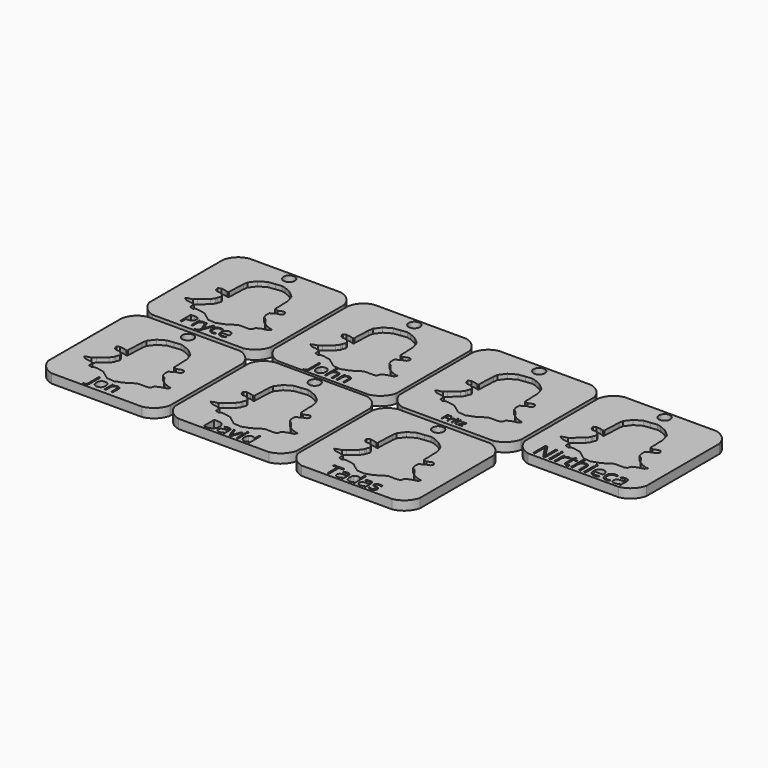
from build123d import *

# Parameters (mm, degrees)
F0_R     = 1.5602718486
F1_DEPTH = 2.54
F0_W     = 0.4165491749
F0_H     = 2.7489035145
F0_W_2   = 0.4850751217
F0_H_2   = 3.2011219496
F2_DEPTH = 1.27


with BuildPart() as f1:
    # F0 (on Top) → F1 (new body)
    with BuildSketch(Plane.XY):
        with BuildLine():
            Line((-70.8376746476, 11.3606358815), (-58.1789253822, 11.3606358815))
            Line((-58.1789253822, 11.3606358815), (-45.6926576544, 11.3606358815))
            ThreePointArc((-45.6926576544, 11.3606358815), (-42.8969714319, 12.8003713157), (-41.3217412719, 15.5220159505))
            Line((-41.3217412719, 15.5220159505), (-41.3217412719, 40.9571273043))
            ThreePointArc((-41.3217412719, 40.9571273043), (-42.8497619053, 43.6115706298), (-45.5290152, 45.0956589718))
            Line((-45.5290152, 45.0956589718), (-70.9290152, 45.0956589718))
            ThreePointArc((-70.9290152, 45.0956589718), (-73.6670388714, 43.720062879), (-75.0617337127, 40.9917182279))
            Line((-75.0617337127, 40.9917182279), (-75.0617337127, 15.503866579))
            ThreePointArc((-75.0617337127, 15.503866579), (-73.5105486534, 12.8604655021), (-70.8376746476, 11.3606358815))
        make_face()
        with BuildLine():
            add(Edge.make_bspline(
                [(-63.4200171323, 16.5564022282), (-62.0189894871, 16.5564022282), (-62.0189894871, 15.4671687026)],
                knots=[0, 0, 0, 1, 1, 1], degree=2))
            add(Edge.make_bspline(
                [(-62.0189894871, 15.4671687026), (-62.0189894871, 14.8992287577), (-62.4064816542, 14.5935723176)],
                knots=[0, 0, 0, 1, 1, 1], degree=2))
            add(Edge.make_bspline(
                [(-62.4064816542, 14.5935723176), (-62.7939738212, 14.2879158775), (-63.5149465755, 14.2879158775)],
                knots=[0, 0, 0, 1, 1, 1], degree=2))
            Line((-63.5149465755, 14.2879158775), (-63.9552227864, 14.2879158775))
            Line((-63.9552227864, 14.2879158775), (-63.9552227864, 12.8173278645))
            Line((-63.9552227864, 12.8173278645), (-64.3897704964, 12.8173278645))
            Line((-64.3897704964, 12.8173278645), (-64.3897704964, 16.5564022282))
            Line((-64.3897704964, 16.5564022282), (-63.4200171323, 16.5564022282))
        make_face(mode=Mode.SUBTRACT)
        with BuildLine():
            add(Edge.make_bspline(
                [(-58.2668214071, 13.2314166428), (-58.2427639866, 13.3276463249), (-58.1789253822, 13.5237709797)],
                knots=[0, 0, 0, 0.7349302513, 0.7349302513, 0.7349302513], degree=2))
            add(Edge.make_bspline(
                [(-58.1789253822, 13.5237709797), (-58.1559004996, 13.5945079141), (-58.1277006713, 13.6782397118)],
                knots=[0.7349302513, 0.7349302513, 0.7349302513, 1, 1, 1], degree=2))
            add(Edge.make_bspline(
                [(-58.1277006713, 13.6782397118), (-58.0213142263, 13.9941256178), (-57.4329153496, 15.620201512)],
                knots=[0, 0, 0, 1, 1, 1], degree=2))
            Line((-57.4329153496, 15.620201512), (-56.9779087079, 15.620201512))
            Line((-56.9779087079, 15.620201512), (-58.1789253822, 12.4381600514))
            Line((-58.1789253822, 12.4381600514), (-58.1825306084, 12.4286081615))
            add(Edge.make_bspline(
                [(-58.1825306084, 12.4286081615), (-58.3617508504, 11.9555976598), (-58.600711173, 11.757146022)],
                knots=[0, 0, 0, 1, 1, 1], degree=2))
            add(Edge.make_bspline(
                [(-58.600711173, 11.757146022), (-58.8396714957, 11.5586943842), (-59.1874733351, 11.5586943842)],
                knots=[0, 0, 0, 1, 1, 1], degree=2))
            add(Edge.make_bspline(
                [(-59.1874733351, 11.5586943842), (-59.3822423652, 11.5586943842), (-59.5712828945, 11.6028856767)],
                knots=[0, 0, 0, 1, 1, 1], degree=2))
            Line((-59.5712828945, 11.6028856767), (-59.5712828945, 11.9425039435))
            add(Edge.make_bspline(
                [(-59.5712828945, 11.9425039435), (-59.4305254441, 11.9122247246), (-59.257033703, 11.9122247246)],
                knots=[0, 0, 0, 1, 1, 1], degree=2))
            add(Edge.make_bspline(
                [(-59.257033703, 11.9122247246), (-58.8192125639, 11.9122247246), (-58.6326271065, 12.4032390862)],
                knots=[0, 0, 0, 1, 1, 1], degree=2))
            Line((-58.6326271065, 12.4032390862), (-58.4763208681, 12.8017790764))
            Line((-58.4763208681, 12.8017790764), (-59.6072906143, 15.620201512))
            Line((-59.6072906143, 15.620201512), (-59.1514656153, 15.620201512))
            Line((-59.1514656153, 15.620201512), (-58.5376976633, 14.021949765))
            add(Edge.make_bspline(
                [(-58.5376976633, 14.021949765), (-58.336381775, 13.4744687518), (-58.2872803388, 13.2314166428)],
                knots=[0, 0, 0, 1, 1, 1], degree=2))
            Line((-58.2872803388, 13.2314166428), (-58.2668214071, 13.2314166428))
        make_face(mode=Mode.SUBTRACT)
        with BuildLine():
            add(Edge.make_bspline(
                [(-60.5050285388, 15.5232261756), (-60.2848904333, 15.67175802), (-60.0213793926, 15.67175802)],
                knots=[0, 0, 0, 1, 1, 1], degree=2))
            add(Edge.make_bspline(
                [(-60.0213793926, 15.67175802), (-59.8347939352, 15.67175802), (-59.6866712694, 15.6406604438)],
                knots=[0, 0, 0, 1, 1, 1], degree=2))
            Line((-59.6866712694, 15.6406604438), (-59.7455929928, 15.2470305972))
            add(Edge.make_bspline(
                [(-59.7455929928, 15.2470305972), (-59.9190847339, 15.2854933888), (-60.0524769688, 15.2854933888)],
                knots=[0, 0, 0, 1, 1, 1], degree=2))
            add(Edge.make_bspline(
                [(-60.0524769688, 15.2854933888), (-60.3929135929, 15.2854933888), (-60.6343289874, 15.0092978104)],
                knots=[0, 0, 0, 1, 1, 1], degree=2))
            add(Edge.make_bspline(
                [(-60.6343289874, 15.0092978104), (-60.8757443818, 14.733102232), (-60.8757443818, 14.3214685255)],
                knots=[0, 0, 0, 1, 1, 1], degree=2))
            Line((-60.8757443818, 14.3214685255), (-60.8757443818, 12.8173278645))
            Line((-60.8757443818, 12.8173278645), (-61.3004718046, 12.8173278645))
            Line((-61.3004718046, 12.8173278645), (-61.3004718046, 15.620201512))
            Line((-61.3004718046, 15.620201512), (-60.9502148933, 15.620201512))
            Line((-60.9502148933, 15.620201512), (-60.9011134572, 15.1013630032))
            Line((-60.9011134572, 15.1013630032), (-60.8806545254, 15.1013630032))
            add(Edge.make_bspline(
                [(-60.8806545254, 15.1013630032), (-60.7251666443, 15.3746943312), (-60.5050285388, 15.5232261756)],
                knots=[0, 0, 0, 1, 1, 1], degree=2))
        make_face(mode=Mode.SUBTRACT)
        with BuildLine():
            add(Edge.make_bspline(
                [(-54.6946919264, 12.9122573077), (-54.9753884698, 12.7657713565), (-55.4025709644, 12.7657713565)],
                knots=[0, 0, 0, 1, 1, 1], degree=2))
            add(Edge.make_bspline(
                [(-55.4025709644, 12.7657713565), (-56.0114287728, 12.7657713565), (-56.3453185387, 13.1405789859)],
                knots=[0, 0, 0, 1, 1, 1], degree=2))
            add(Edge.make_bspline(
                [(-56.3453185387, 13.1405789859), (-56.6792083046, 13.5153866152), (-56.6792083046, 14.201170007)],
                knots=[0, 0, 0, 1, 1, 1], degree=2))
            add(Edge.make_bspline(
                [(-56.6792083046, 14.201170007), (-56.6792083046, 14.9041389013), (-56.3399992164, 15.2879484607)],
                knots=[0, 0, 0, 1, 1, 1], degree=2))
            add(Edge.make_bspline(
                [(-56.3399992164, 15.2879484607), (-56.0007901283, 15.67175802), (-55.3747468172, 15.67175802)],
                knots=[0, 0, 0, 1, 1, 1], degree=2))
            add(Edge.make_bspline(
                [(-55.3747468172, 15.67175802), (-55.1726125717, 15.67175802), (-54.9704783261, 15.6279759061)],
                knots=[0, 0, 0, 1, 1, 1], degree=2))
            add(Edge.make_bspline(
                [(-54.9704783261, 15.6279759061), (-54.7683440806, 15.5841937922), (-54.6537740629, 15.5252720688)],
                knots=[0, 0, 0, 1, 1, 1], degree=2))
            Line((-54.6537740629, 15.5252720688), (-54.7838928687, 15.1651948703))
            add(Edge.make_bspline(
                [(-54.7838928687, 15.1651948703), (-54.9246503191, 15.2216615218), (-55.0907768447, 15.258487599)],
                knots=[0, 0, 0, 1, 1, 1], degree=2))
            add(Edge.make_bspline(
                [(-55.0907768447, 15.258487599), (-55.2569033704, 15.2953136761), (-55.3845671044, 15.2953136761)],
                knots=[0, 0, 0, 1, 1, 1], degree=2))
            add(Edge.make_bspline(
                [(-55.3845671044, 15.2953136761), (-56.2389320936, 15.2953136761), (-56.2389320936, 14.2060801506)],
                knots=[0, 0, 0, 1, 1, 1], degree=2))
            add(Edge.make_bspline(
                [(-56.2389320936, 14.2060801506), (-56.2389320936, 13.6896967136), (-56.0306601686, 13.4135011352)],
                knots=[0, 0, 0, 1, 1, 1], degree=2))
            add(Edge.make_bspline(
                [(-56.0306601686, 13.4135011352), (-55.8223882435, 13.1373055568), (-55.4132096089, 13.1373055568)],
                knots=[0, 0, 0, 1, 1, 1], degree=2))
            add(Edge.make_bspline(
                [(-55.4132096089, 13.1373055568), (-55.0629526976, 13.1373055568), (-54.6946919264, 13.2878832943)],
                knots=[0, 0, 0, 1, 1, 1], degree=2))
            Line((-54.6946919264, 13.2878832943), (-54.6946919264, 12.9122573077))
        make_face(mode=Mode.SUBTRACT)
        with BuildLine():
            add(Edge.make_bspline(
                [(-52.3607369942, 12.8083259345), (-52.5612345252, 12.7657713565), (-52.8452044976, 12.7657713565)],
                knots=[0, 0, 0, 1, 1, 1], degree=2))
            add(Edge.make_bspline(
                [(-52.8452044976, 12.7657713565), (-53.4663376651, 12.7657713565), (-53.8260056849, 13.1446707722)],
                knots=[0, 0, 0, 1, 1, 1], degree=2))
            add(Edge.make_bspline(
                [(-53.8260056849, 13.1446707722), (-54.1856737048, 13.5235701879), (-54.1856737048, 14.1954415061)],
                knots=[0, 0, 0, 1, 1, 1], degree=2))
            add(Edge.make_bspline(
                [(-54.1856737048, 14.1954415061), (-54.1856737048, 14.8738596824), (-53.8517839389, 15.2728088512)],
                knots=[0, 0, 0, 1, 1, 1], degree=2))
            add(Edge.make_bspline(
                [(-53.8517839389, 15.2728088512), (-53.517894173, 15.67175802), (-52.9548643717, 15.67175802)],
                knots=[0, 0, 0, 1, 1, 1], degree=2))
            add(Edge.make_bspline(
                [(-52.9548643717, 15.67175802), (-52.4286606475, 15.67175802), (-52.1217766715, 15.3251837164)],
                knots=[0, 0, 0, 1, 1, 1], degree=2))
            add(Edge.make_bspline(
                [(-52.1217766715, 15.3251837164), (-51.8148926955, 14.9786094128), (-51.8148926955, 14.4106694679)],
                knots=[0, 0, 0, 1, 1, 1], degree=2))
            Line((-51.8148926955, 14.4106694679), (-51.8148926955, 14.1422482836))
            Line((-51.8148926955, 14.1422482836), (-53.7453974939, 14.1422482836))
            add(Edge.make_bspline(
                [(-53.7453974939, 14.1422482836), (-53.7323037776, 13.6487788501), (-53.4957985268, 13.3930422035)],
                knots=[0, 0, 0, 1, 1, 1], degree=2))
            add(Edge.make_bspline(
                [(-53.4957985268, 13.3930422035), (-53.2592932759, 13.1373055568), (-52.8296557095, 13.1373055568)],
                knots=[0, 0, 0, 1, 1, 1], degree=2))
            add(Edge.make_bspline(
                [(-52.8296557095, 13.1373055568), (-52.3771041395, 13.1373055568), (-51.9351912141, 13.326346086)],
                knots=[0, 0, 0, 1, 1, 1], degree=2))
            Line((-51.9351912141, 13.326346086), (-51.9351912141, 12.9474466703))
            add(Edge.make_bspline(
                [(-51.9351912141, 12.9474466703), (-52.1602394632, 12.8508805125), (-52.3607369942, 12.8083259345)],
                knots=[0, 0, 0, 1, 1, 1], degree=2))
        make_face(mode=Mode.SUBTRACT)
        Polygon((-64.5831264968, 30.0570140501), (-64.6589176566, 30.3048104431), (-64.4690111618, 34.8625764245), (-64.2791046669, 36.0969661146), (-62.9497541504, 37.877352767), (-60.9557334283, 39.0167917361), (-59.1041438404, 39.2541685387), (-57.3475049737, 39.4678177665), (-56.3030167257, 39.2066931782), (-54.5938532195, 38.4470671988), (-53.8342272402, 37.877352767), (-52.7422636317, 36.9278152402), (-52.362450642, 36.0969661146), (-51.9351622918, 34.5302387954), (-51.9351622918, 33.034724517), (-51.840206518, 31.8003348269), (-51.840206518, 30.6134103919), (-51.840206518, 30.1386466812), (-50.9856247649, 29.8063090521), (-49.7037546616, 30.2810727628), (-49.1815105376, 30.2810727628), (-48.801697548, 29.8063090521), (-48.801697548, 29.2945493228), (-49.141770892, 28.8931309009), (-49.734338778, 28.6255186196), (-50.1357571999, 28.6255186196), (-50.823907397, 28.1285229393), (-51.5694009175, 27.7653333996), (-51.5694009175, 27.2109994486), (-51.5694009175, 26.4846203693), (-51.2826691423, 25.6244351493), (-50.3651405989, 24.955404446), (-49.2564575388, 23.4261784174), (-48.3911920396, 22.7952561539), (-47.650783851, 22.5086549267), (-46.7332553076, 22.1645747754), (-46.198030745, 22.1645747754), (-46.4645777568, 21.7990243003), (-46.5803347259, 21.514663566), (-47.0390964712, 21.3426285431), (-48.3198145543, 21.0176678857), (-49.103536957, 20.654478346), (-49.5431893139, 20.425094947), (-49.7343438307, 19.5840292209), (-50.3651405989, 19.2549184939), (-52.2186451678, 19.2549184939), (-53.1681776419, 19.2424956407), (-54.3656050664, 18.6177520941), (-54.7586476941, 18.2454827533), (-55.6826779645, 17.7633809269), (-56.2541619725, 17.4858567739), (-57.4410813548, 17.1060437842), (-57.8540122926, 16.8906019685), (-58.1789253822, 16.9231915715), (-59.0552890873, 17.0110930632), (-59.9573462009, 17.0585684237), (-60.8572082395, 17.7147173107), (-61.9007541664, 18.4756356171), (-62.473611047, 18.9576333721), (-63.3994058409, 19.1475449196), (-64.5625875429, 19.3849217223), (-65.4171667696, 19.3849217223), (-65.7969797593, 19.0051087326), (-66.8414680073, 19.361184042), (-66.8414680073, 20.654478346), (-68.0283873895, 21.0940852285), (-69.4289484205, 21.283996776), (-70.3230021459, 21.935910438), (-69.7115546332, 22.2549259205), (-68.6218445543, 22.4946487858), (-67.8622185749, 23.1830617244), (-65.7257667185, 24.955404446), (-65.0474260791, 25.885700912), (-64.9186628523, 26.4114771893), (-64.5388498626, 27.3135393557), (-64.8821209506, 27.9714768678), (-65.8581243732, 28.6831454703), (-66.8889458942, 28.6831454703), (-67.3705666986, 29.0343270306), (-67.6723120801, 29.6873781202), (-67.6723120801, 29.9722302833), (-66.9738093314, 30.336665802), (-65.7969822857, 30.1858795112), (-64.8821209506, 29.9010172425), align=None, mode=Mode.SUBTRACT)
        with Locations((-58.3071684778, 43.0780872703)):
            Circle(F0_R, mode=Mode.SUBTRACT)
    extrude(amount=F1_DEPTH)

    # F0 (on Top) → F2 (join)
    with BuildSketch(Plane.XY):
        Polygon((-64.4690111618, 34.8625764245), (-64.6589176566, 30.3048104431), (-64.5831264968, 30.0570140501), (-64.8821209506, 29.9010172425), (-65.7969822857, 30.1858795112), (-66.9738093314, 30.336665802), (-67.6723120801, 29.9722302833), (-67.6723120801, 29.6873781202), (-67.3705666986, 29.0343270306), (-66.8889458942, 28.6831454703), (-65.8581243732, 28.6831454703), (-64.8821209506, 27.9714768678), (-64.5388498626, 27.3135393557), (-64.9186628523, 26.4114771893), (-65.0474260791, 25.885700912), (-65.7257667185, 24.955404446), (-67.8622185749, 23.1830617244), (-68.6218445543, 22.4946487858), (-69.7115546332, 22.2549259205), (-70.3230021459, 21.935910438), (-69.4289484205, 21.283996776), (-68.0283873895, 21.0940852285), (-66.8414680073, 20.654478346), (-66.8414680073, 19.361184042), (-65.7969797593, 19.0051087326), (-65.4171667696, 19.3849217223), (-64.5625875429, 19.3849217223), (-63.3994058409, 19.1475449196), (-62.473611047, 18.9576333721), (-61.9007541664, 18.4756356171), (-60.8572082395, 17.7147173107), (-59.9573462009, 17.0585684237), (-59.0552890873, 17.0110930632), (-58.1789253822, 16.9231915715), (-57.8540122926, 16.8906019685), (-57.4410813548, 17.1060437842), (-56.2541619725, 17.4858567739), (-55.6826779645, 17.7633809269), (-54.7586476941, 18.2454827533), (-54.3656050664, 18.6177520941), (-53.1681776419, 19.2424956407), (-52.2186451678, 19.2549184939), (-50.3651405989, 19.2549184939), (-49.7343438307, 19.5840292209), (-49.5431893139, 20.425094947), (-49.103536957, 20.654478346), (-48.3198145543, 21.0176678857), (-47.0390964712, 21.3426285431), (-46.5803347259, 21.514663566), (-46.4645777568, 21.7990243003), (-46.198030745, 22.1645747754), (-46.7332553076, 22.1645747754), (-47.650783851, 22.5086549267), (-48.3911920396, 22.7952561539), (-49.2564575388, 23.4261784174), (-50.3651405989, 24.955404446), (-51.2826691423, 25.6244351493), (-51.5694009175, 26.4846203693), (-51.5694009175, 27.2109994486), (-51.5694009175, 27.7653333996), (-50.823907397, 28.1285229393), (-50.1357571999, 28.6255186196), (-49.734338778, 28.6255186196), (-49.141770892, 28.8931309009), (-48.801697548, 29.2945493228), (-48.801697548, 29.8063090521), (-49.1815105376, 30.2810727628), (-49.7037546616, 30.2810727628), (-50.9856247649, 29.8063090521), (-51.840206518, 30.1386466812), (-51.840206518, 30.6134103919), (-51.840206518, 31.8003348269), (-51.9351622918, 33.034724517), (-51.9351622918, 34.5302387954), (-52.362450642, 36.0969661146), (-52.7422636317, 36.9278152402), (-53.8342272402, 37.877352767), (-54.5938532195, 38.4470671988), (-56.3030167257, 39.2066931782), (-57.3475049737, 39.4678177665), (-59.1041438404, 39.2541685387), (-60.9557334283, 39.0167917361), (-62.9497541504, 37.877352767), (-64.2791046669, 36.0969661146), align=None)
    extrude(amount=F2_DEPTH)


with BuildPart() as f1b:
    # F0 (on Top) → F1, piece 2 (new body)
    with BuildSketch(Plane.XY):
        with BuildLine():
            Line((-70.8376746476, -23.7765275746), (-58.1789253822, -23.7765275746))
            Line((-58.1789253822, -23.7765275746), (-45.6926576544, -23.7765275746))
            ThreePointArc((-45.6926576544, -23.7765275746), (-42.8969714319, -22.3367921404), (-41.3217412719, -19.6151475056))
            Line((-41.3217412719, -19.6151475056), (-41.3217412719, 5.8199638482))
            ThreePointArc((-41.3217412719, 5.8199638482), (-42.8497619053, 8.4744071736), (-45.5290152, 9.9584955157))
            Line((-45.5290152, 9.9584955157), (-70.9290152, 9.9584955157))
            ThreePointArc((-70.9290152, 9.9584955157), (-73.6670388714, 8.5828994229), (-75.0617337127, 5.8545547718))
            Line((-75.0617337127, 5.8545547718), (-75.0617337127, -19.6332968771))
            ThreePointArc((-75.0617337127, -19.6332968771), (-73.5105486534, -22.276697954), (-70.8376746476, -23.7765275746))
        make_face()
        with BuildLine():
            add(Edge.make_bspline(
                [(-61.5135747709, -23.2130668772), (-61.7589163024, -23.4800802439), (-62.2193405765, -23.4800802439)],
                knots=[0, 0, 0, 1, 1, 1], degree=2))
            add(Edge.make_bspline(
                [(-62.2193405765, -23.4800802439), (-62.4589574723, -23.4800802439), (-62.597166535, -23.4113846151)],
                knots=[0, 0, 0, 1, 1, 1], degree=2))
            Line((-62.597166535, -23.4113846151), (-62.597166535, -23.0409189026))
            add(Edge.make_bspline(
                [(-62.597166535, -23.0409189026), (-62.4156138017, -23.0916228191), (-62.2193405765, -23.0916228191)],
                knots=[0, 0, 0, 1, 1, 1], degree=2))
            add(Edge.make_bspline(
                [(-62.2193405765, -23.0916228191), (-61.965820994, -23.0916228191), (-61.8341543721, -22.9382843619)],
                knots=[0, 0, 0, 1, 1, 1], degree=2))
            add(Edge.make_bspline(
                [(-61.8341543721, -22.9382843619), (-61.7024877502, -22.7849459047), (-61.7024877502, -22.4962607026)],
                knots=[0, 0, 0, 1, 1, 1], degree=2))
            Line((-61.7024877502, -22.4962607026), (-61.7024877502, -18.7597091778))
            Line((-61.7024877502, -18.7597091778), (-61.2682332394, -18.7597091778))
            Line((-61.2682332394, -18.7597091778), (-61.2682332394, -22.460277278))
            add(Edge.make_bspline(
                [(-61.2682332394, -22.460277278), (-61.2682332394, -22.9460535104), (-61.5135747709, -23.2130668772)],
                knots=[0, 0, 0, 1, 1, 1], degree=2))
        make_face(mode=Mode.SUBTRACT)
        with BuildLine():
            add(Edge.make_bspline(
                [(-58.2697508218, -20.0350762391), (-58.2208917725, -20.0902806194), (-58.1789253822, -20.1509616934)],
                knots=[0, 0, 0, 0.1410723108, 0.1410723108, 0.1410723108], degree=2))
            add(Edge.make_bspline(
                [(-58.1789253822, -20.1509616934), (-57.9234103599, -20.5204222514), (-57.9234103599, -21.0929071424)],
                knots=[0.1410723108, 0.1410723108, 0.1410723108, 1, 1, 1], degree=2))
            add(Edge.make_bspline(
                [(-57.9234103599, -21.0929071424), (-57.9234103599, -21.6829429343), (-58.1789253822, -22.0501987246)],
                knots=[0, 0, 0, 0.8609630657, 0.8609630657, 0.8609630657], degree=2))
            add(Edge.make_bspline(
                [(-58.1789253822, -22.0501987246), (-58.2201885058, -22.1095068659), (-58.2681152116, -22.1630051223)],
                knots=[0.8609630657, 0.8609630657, 0.8609630657, 1, 1, 1], degree=2))
            add(Edge.make_bspline(
                [(-58.2681152116, -22.1630051223), (-58.6128200634, -22.5477824242), (-59.2212670615, -22.5477824242)],
                knots=[0, 0, 0, 1, 1, 1], degree=2))
            add(Edge.make_bspline(
                [(-59.2212670615, -22.5477824242), (-59.5974574098, -22.5477824242), (-59.8885960272, -22.3711365215)],
                knots=[0, 0, 0, 1, 1, 1], degree=2))
            add(Edge.make_bspline(
                [(-59.8885960272, -22.3711365215), (-60.1797346446, -22.1944906189), (-60.338388835, -21.8649151615)],
                knots=[0, 0, 0, 1, 1, 1], degree=2))
            add(Edge.make_bspline(
                [(-60.338388835, -21.8649151615), (-60.4970430254, -21.5353397042), (-60.4970430254, -21.0929071424)],
                knots=[0, 0, 0, 1, 1, 1], degree=2))
            add(Edge.make_bspline(
                [(-60.4970430254, -21.0929071424), (-60.4970430254, -20.4084042695), (-60.1543826864, -20.0260803829)],
                knots=[0, 0, 0, 1, 1, 1], degree=2))
            add(Edge.make_bspline(
                [(-60.1543826864, -20.0260803829), (-59.8117223474, -19.6437564963), (-59.2032753492, -19.6437564963)],
                knots=[0, 0, 0, 1, 1, 1], degree=2))
            add(Edge.make_bspline(
                [(-59.2032753492, -19.6437564963), (-58.6160912838, -19.6437564963), (-58.2697508218, -20.0350762391)],
                knots=[0, 0, 0, 1, 1, 1], degree=2))
        make_face(mode=Mode.SUBTRACT)
        with BuildLine():
            Line((-54.8378316986, -22.4962607026), (-55.2622725481, -22.4962607026))
            Line((-55.2622725481, -22.4962607026), (-55.2622725481, -20.6840045899))
            add(Edge.make_bspline(
                [(-55.2622725481, -20.6840045899), (-55.2622725481, -20.342162056), (-55.4180644206, -20.1732853018)],
                knots=[0, 0, 0, 1, 1, 1], degree=2))
            add(Edge.make_bspline(
                [(-55.4180644206, -20.1732853018), (-55.5738562931, -20.0044085476), (-55.9067029709, -20.0044085476)],
                knots=[0, 0, 0, 1, 1, 1], degree=2))
            add(Edge.make_bspline(
                [(-55.9067029709, -20.0044085476), (-56.3458643123, -20.0044085476), (-56.5503155885, -20.2419809306)],
                knots=[0, 0, 0, 1, 1, 1], degree=2))
            add(Edge.make_bspline(
                [(-56.5503155885, -20.2419809306), (-56.7547668648, -20.4795533136), (-56.7547668648, -21.0266649289)],
                knots=[0, 0, 0, 1, 1, 1], degree=2))
            Line((-56.7547668648, -21.0266649289), (-56.7547668648, -22.4962607026))
            Line((-56.7547668648, -22.4962607026), (-57.1792077143, -22.4962607026))
            Line((-57.1792077143, -22.4962607026), (-57.1792077143, -19.6952782179))
            Line((-57.1792077143, -19.6952782179), (-56.83409396, -19.6952782179))
            Line((-56.83409396, -19.6952782179), (-56.7653983312, -20.0788288122))
            Line((-56.7653983312, -20.0788288122), (-56.7449532035, -20.0788288122))
            add(Edge.make_bspline(
                [(-56.7449532035, -20.0788288122), (-56.6141043867, -19.8719241206), (-56.378985419, -19.7578403085)],
                knots=[0, 0, 0, 1, 1, 1], degree=2))
            add(Edge.make_bspline(
                [(-56.378985419, -19.7578403085), (-56.1438664513, -19.6437564963), (-55.8551812493, -19.6437564963)],
                knots=[0, 0, 0, 1, 1, 1], degree=2))
            add(Edge.make_bspline(
                [(-55.8551812493, -19.6437564963), (-55.3489598893, -19.6437564963), (-55.0933957939, -19.8878713202)],
                knots=[0, 0, 0, 1, 1, 1], degree=2))
            add(Edge.make_bspline(
                [(-55.0933957939, -19.8878713202), (-54.8378316986, -20.131986144), (-54.8378316986, -20.669284098)],
                knots=[0, 0, 0, 1, 1, 1], degree=2))
            Line((-54.8378316986, -20.669284098), (-54.8378316986, -22.4962607026))
        make_face(mode=Mode.SUBTRACT)
        Polygon((-64.5831264968, -5.0801494061), (-64.6589176566, -4.8323530131), (-64.4690111618, -0.2745870316), (-64.2791046669, 0.9598026585), (-62.9497541504, 2.7401893109), (-60.9557334283, 3.8796282799), (-59.1041438404, 4.1170050826), (-57.3475049737, 4.3306543104), (-56.3030167257, 4.069529722), (-54.5938532195, 3.3099037427), (-53.8342272402, 2.7401893109), (-52.7422636317, 1.790651784), (-52.362450642, 0.9598026585), (-51.9351622918, -0.6069246607), (-51.9351622918, -2.1024389392), (-51.840206518, -3.3368286292), (-51.840206518, -4.5237530642), (-51.840206518, -4.9985167749), (-50.9856247649, -5.3308544041), (-49.7037546616, -4.8560906933), (-49.1815105376, -4.8560906933), (-48.801697548, -5.3308544041), (-48.801697548, -5.8426141333), (-49.141770892, -6.2440325552), (-49.734338778, -6.5116448365), (-50.1357571999, -6.5116448365), (-50.823907397, -7.0086405168), (-51.5694009175, -7.3718300565), (-51.5694009175, -7.9261640075), (-51.5694009175, -8.6525430869), (-51.2826691423, -9.5127283069), (-50.3651405989, -10.1817590101), (-49.2564575388, -11.7109850388), (-48.3911920396, -12.3419073022), (-47.650783851, -12.6285085294), (-46.7332553076, -12.9725886807), (-46.198030745, -12.9725886807), (-46.4645777568, -13.3381391558), (-46.5803347259, -13.6224998901), (-47.0390964712, -13.794534913), (-48.3198145543, -14.1194955704), (-49.103536957, -14.4826851101), (-49.5431893139, -14.7120685091), (-49.7343438307, -15.5531342352), (-50.3651405989, -15.8822449622), (-52.2186451678, -15.8822449622), (-53.1681776419, -15.8946678154), (-54.3656050664, -16.519411362), (-54.7586476941, -16.8916807029), (-55.6826779645, -17.3737825292), (-56.2541619725, -17.6513066822), (-57.4410813548, -18.0311196719), (-57.8540122926, -18.2465614876), (-58.1789253822, -18.2139718846), (-59.0552890873, -18.1260703929), (-59.9573462009, -18.0785950324), (-60.8572082395, -17.4224461454), (-61.9007541664, -16.661527839), (-62.473611047, -16.1795300841), (-63.3994058409, -15.9896185365), (-64.5625875429, -15.7522417339), (-65.4171667696, -15.7522417339), (-65.7969797593, -16.1320547235), (-66.8414680073, -15.7759794141), (-66.8414680073, -14.4826851101), (-68.0283873895, -14.0430782276), (-69.4289484205, -13.8531666801), (-70.3230021459, -13.2012530182), (-69.7115546332, -12.8822375356), (-68.6218445543, -12.6425146703), (-67.8622185749, -11.9541017317), (-65.7257667185, -10.1817590101), (-65.0474260791, -9.2514625441), (-64.9186628523, -8.7256862668), (-64.5388498626, -7.8236241005), (-64.8821209506, -7.1656865883), (-65.8581243732, -6.4540179858), (-66.8889458942, -6.4540179858), (-67.3705666986, -6.1028364255), (-67.6723120801, -5.449785336), (-67.6723120801, -5.1649331728), (-66.9738093314, -4.8004976541), (-65.7969822857, -4.951283945), (-64.8821209506, -5.2361462136), align=None, mode=Mode.SUBTRACT)
        with Locations((-58.3071684778, 7.9409238141)):
            Circle(F0_R, mode=Mode.SUBTRACT)
    extrude(amount=F1_DEPTH)


with BuildPart() as f1c:
    # F0 (on Top) → F1, piece 3 (new body)
    with BuildSketch(Plane.XY):
        with BuildLine():
            Line((-36.0487467747, -23.2375618875), (-23.3899975093, -23.2375618875))
            Line((-23.3899975093, -23.2375618875), (-10.9037297814, -23.2375618875))
            ThreePointArc((-10.9037297814, -23.2375618875), (-8.108043559, -21.7978264532), (-6.532813399, -19.0761818184))
            Line((-6.532813399, -19.0761818184), (-6.532813399, 6.3589295354))
            ThreePointArc((-6.532813399, 6.3589295354), (-8.0608340324, 9.0133728608), (-10.740087327, 10.4974612029))
            Line((-10.740087327, 10.4974612029), (-36.140087327, 10.4974612029))
            ThreePointArc((-36.140087327, 10.4974612029), (-38.8781109984, 9.1218651101), (-40.2728058398, 6.393520459))
            Line((-40.2728058398, 6.393520459), (-40.2728058398, -19.09433119))
            ThreePointArc((-40.2728058398, -19.09433119), (-38.7216207804, -21.7377322668), (-36.0487467747, -23.2375618875))
        make_face()
        with BuildLine():
            add(Edge.make_bspline(
                [(-27.1446036091, -19.3111444662), (-26.6706685652, -19.7850795101), (-26.6706685652, -20.6358350503)],
                knots=[0, 0, 0, 1, 1, 1], degree=2))
            add(Edge.make_bspline(
                [(-26.6706685652, -20.6358350503), (-26.6706685652, -21.5435751597), (-27.1634646989, -22.0239310001)],
                knots=[0, 0, 0, 1, 1, 1], degree=2))
            add(Edge.make_bspline(
                [(-27.1634646989, -22.0239310001), (-27.6562608326, -22.5042868406), (-28.5816581325, -22.5042868406)],
                knots=[0, 0, 0, 1, 1, 1], degree=2))
            Line((-28.5816581325, -22.5042868406), (-29.5977491834, -22.5042868406))
            Line((-29.5977491834, -22.5042868406), (-29.5977491834, -18.8372094223))
            Line((-29.5977491834, -18.8372094223), (-28.4741097906, -18.8372094223))
            add(Edge.make_bspline(
                [(-28.4741097906, -18.8372094223), (-27.618538653, -18.8372094223), (-27.1446036091, -19.3111444662)],
                knots=[0, 0, 0, 1, 1, 1], degree=2))
        make_face(mode=Mode.SUBTRACT)
        with BuildLine():
            Line((-23.9161468538, -22.5042868406), (-24.2251476868, -22.5042868406))
            Line((-24.2251476868, -22.5042868406), (-24.3078154421, -22.1126182522))
            Line((-24.3078154421, -22.1126182522), (-24.3278804313, -22.1126182522))
            add(Edge.make_bspline(
                [(-24.3278804313, -22.1126182522), (-24.5333459202, -22.3710553126), (-24.7376075099, -22.4629529629)],
                knots=[0, 0, 0, 1, 1, 1], degree=2))
            add(Edge.make_bspline(
                [(-24.7376075099, -22.4629529629), (-24.9418690995, -22.5548506132), (-25.2484621338, -22.5548506132)],
                knots=[0, 0, 0, 1, 1, 1], degree=2))
            add(Edge.make_bspline(
                [(-25.2484621338, -22.5548506132), (-25.656985313, -22.5548506132), (-25.8889365877, -22.3437669273)],
                knots=[0, 0, 0, 1, 1, 1], degree=2))
            add(Edge.make_bspline(
                [(-25.8889365877, -22.3437669273), (-26.1208878623, -22.1326832414), (-26.1208878623, -21.7442250513)],
                knots=[0, 0, 0, 1, 1, 1], degree=2))
            add(Edge.make_bspline(
                [(-26.1208878623, -21.7442250513), (-26.1208878623, -20.9119293011), (-24.7893751819, -20.8717993228)],
                knots=[0, 0, 0, 1, 1, 1], degree=2))
            Line((-24.7893751819, -20.8717993228), (-24.3230648339, -20.856549931))
            Line((-24.3230648339, -20.856549931), (-24.3230648339, -20.6855962234))
            add(Edge.make_bspline(
                [(-24.3230648339, -20.6855962234), (-24.3230648339, -20.3621485982), (-24.4619145588, -20.2080494815)],
                knots=[0, 0, 0, 1, 1, 1], degree=2))
            add(Edge.make_bspline(
                [(-24.4619145588, -20.2080494815), (-24.6007642838, -20.0539503648), (-24.9073573181, -20.0539503648)],
                knots=[0, 0, 0, 1, 1, 1], degree=2))
            add(Edge.make_bspline(
                [(-24.9073573181, -20.0539503648), (-25.2508699325, -20.0539503648), (-25.6842736983, -20.2642314511)],
                knots=[0, 0, 0, 1, 1, 1], degree=2))
            Line((-25.6842736983, -20.2642314511), (-25.8126896289, -19.9455994233))
            add(Edge.make_bspline(
                [(-25.8126896289, -19.9455994233), (-25.6096319386, -19.8356432827), (-25.3676481694, -19.7730405166)],
                knots=[0, 0, 0, 1, 1, 1], degree=2))
            add(Edge.make_bspline(
                [(-25.3676481694, -19.7730405166), (-25.1256644001, -19.7104377504), (-24.881674132, -19.7104377504)],
                knots=[0, 0, 0, 1, 1, 1], degree=2))
            add(Edge.make_bspline(
                [(-24.881674132, -19.7104377504), (-24.3904831974, -19.7104377504), (-24.1533150256, -19.9283435326)],
                knots=[0, 0, 0, 1, 1, 1], degree=2))
            add(Edge.make_bspline(
                [(-24.1533150256, -19.9283435326), (-23.9161468538, -20.1462493149), (-23.9161468538, -20.6278090546)],
                knots=[0, 0, 0, 1, 1, 1], degree=2))
            Line((-23.9161468538, -20.6278090546), (-23.9161468538, -22.5042868406))
        make_face(mode=Mode.SUBTRACT)
        with BuildLine():
            Line((-23.5004002785, -19.7553833261), (-23.3899975093, -19.7553833261))
            Line((-23.3899975093, -19.7553833261), (-23.0541549196, -19.7553833261))
            Line((-23.0541549196, -19.7553833261), (-22.4618364397, -21.3854630452))
            add(Edge.make_bspline(
                [(-22.4618364397, -21.3854630452), (-22.2611865481, -21.9577165359), (-22.2258721672, -22.127867644)],
                knots=[0, 0, 0, 1, 1, 1], degree=2))
            Line((-22.2258721672, -22.127867644), (-22.2058071781, -22.127867644))
            add(Edge.make_bspline(
                [(-22.2058071781, -22.127867644), (-22.1785187928, -21.9954387155), (-22.0316430722, -21.5776856413)],
                knots=[0, 0, 0, 1, 1, 1], degree=2))
            add(Edge.make_bspline(
                [(-22.0316430722, -21.5776856413), (-21.8847673516, -21.1599325671), (-21.3735114279, -19.7553833261)],
                knots=[0, 0, 0, 1, 1, 1], degree=2))
            Line((-21.3735114279, -19.7553833261), (-20.927266069, -19.7553833261))
            Line((-20.927266069, -19.7553833261), (-21.9706455052, -22.5042868406))
            Line((-21.9706455052, -22.5042868406), (-22.4570208423, -22.5042868406))
            Line((-22.4570208423, -22.5042868406), (-23.3899975093, -20.0462521603))
            Line((-23.3899975093, -20.0462521603), (-23.5004002785, -19.7553833261))
        make_face(mode=Mode.SUBTRACT)
        with Locations((-20.2775617201, -21.1298350833)):
            Rectangle(F0_W, F0_H, mode=Mode.SUBTRACT)
        with BuildLine():
            Line((-17.2601886508, -22.5042868406), (-17.3155680208, -22.1358936396))
            Line((-17.3155680208, -22.1358936396), (-17.3380408087, -22.1358936396))
            add(Edge.make_bspline(
                [(-17.3380408087, -22.1358936396), (-17.626174053, -22.5548506132), (-18.2008353424, -22.5548506132)],
                knots=[0, 0, 0, 1, 1, 1], degree=2))
            add(Edge.make_bspline(
                [(-18.2008353424, -22.5548506132), (-18.7401822509, -22.5548506132), (-19.0399531889, -22.1860561125)],
                knots=[0, 0, 0, 1, 1, 1], degree=2))
            add(Edge.make_bspline(
                [(-19.0399531889, -22.1860561125), (-19.3397241269, -21.8172616118), (-19.3397241269, -21.1374597792)],
                knots=[0, 0, 0, 1, 1, 1], degree=2))
            add(Edge.make_bspline(
                [(-19.3397241269, -21.1374597792), (-19.3397241269, -20.4576579466), (-19.0387492896, -20.08123875)],
                knots=[0, 0, 0, 1, 1, 1], degree=2))
            add(Edge.make_bspline(
                [(-19.0387492896, -20.08123875), (-18.7377744522, -19.7048195534), (-18.2008353424, -19.7048195534)],
                knots=[0, 0, 0, 1, 1, 1], degree=2))
            add(Edge.make_bspline(
                [(-18.2008353424, -19.7048195534), (-17.6414234447, -19.7048195534), (-17.3428564061, -20.1117375335)],
                knots=[0, 0, 0, 1, 1, 1], degree=2))
            Line((-17.3428564061, -20.1117375335), (-17.3099498239, -20.1117375335))
            Line((-17.3099498239, -20.1117375335), (-17.3276070143, -19.9134954407))
            Line((-17.3276070143, -19.9134954407), (-17.3380408087, -19.7200689452))
            Line((-17.3380408087, -19.7200689452), (-17.3380408087, -18.6012451498))
            Line((-17.3380408087, -18.6012451498), (-16.9214916338, -18.6012451498))
            Line((-16.9214916338, -18.6012451498), (-16.9214916338, -22.5042868406))
            Line((-16.9214916338, -22.5042868406), (-17.2601886508, -22.5042868406))
        make_face(mode=Mode.SUBTRACT)
        with BuildLine():
            add(Edge.make_bspline(
                [(-20.4509232264, -19.2200494154), (-20.5211506885, -19.1510258527), (-20.5211506885, -19.0105709286)],
                knots=[0, 0, 0, 1, 1, 1], degree=2))
            add(Edge.make_bspline(
                [(-20.5211506885, -19.0105709286), (-20.5211506885, -18.8677082058), (-20.4509232264, -18.8010924418)],
                knots=[0, 0, 0, 1, 1, 1], degree=2))
            add(Edge.make_bspline(
                [(-20.4509232264, -18.8010924418), (-20.3806957644, -18.7344766778), (-20.2747526216, -18.7344766778)],
                knots=[0, 0, 0, 1, 1, 1], degree=2))
            add(Edge.make_bspline(
                [(-20.2747526216, -18.7344766778), (-20.1744276759, -18.7344766778), (-20.1017924151, -18.8022963412)],
                knots=[0, 0, 0, 1, 1, 1], degree=2))
            add(Edge.make_bspline(
                [(-20.1017924151, -18.8022963412), (-20.0291571544, -18.8701160045), (-20.0291571544, -19.0105709286)],
                knots=[0, 0, 0, 1, 1, 1], degree=2))
            add(Edge.make_bspline(
                [(-20.0291571544, -19.0105709286), (-20.0291571544, -19.1510258527), (-20.1017924151, -19.2200494154)],
                knots=[0, 0, 0, 1, 1, 1], degree=2))
            add(Edge.make_bspline(
                [(-20.1017924151, -19.2200494154), (-20.1744276759, -19.2890729781), (-20.2747526216, -19.2890729781)],
                knots=[0, 0, 0, 1, 1, 1], degree=2))
            add(Edge.make_bspline(
                [(-20.2747526216, -19.2890729781), (-20.3806957644, -19.2890729781), (-20.4509232264, -19.2200494154)],
                knots=[0, 0, 0, 1, 1, 1], degree=2))
        make_face(mode=Mode.SUBTRACT)
        Polygon((-29.7941986239, -4.5411837189), (-29.8699897837, -4.2933873259), (-29.6800832888, 0.2643786556), (-29.490176794, 1.4987683456), (-28.1608262774, 3.2791549981), (-26.1668055553, 4.4185939671), (-24.3152159675, 4.6559707697), (-22.5585771007, 4.8696199975), (-21.5140888528, 4.6084954092), (-19.8049253466, 3.8488694299), (-19.0452993672, 3.2791549981), (-17.9533357587, 2.3296174712), (-17.5735227691, 1.4987683456), (-17.1462344189, -0.0679589736), (-17.1462344189, -1.563473252), (-17.0512786451, -2.7978629421), (-17.0512786451, -3.984787377), (-17.0512786451, -4.4595510878), (-16.196696892, -4.7918887169), (-14.9148267887, -4.3171250062), (-14.3925826647, -4.3171250062), (-14.012769675, -4.7918887169), (-14.012769675, -5.3036484461), (-14.352843019, -5.7050668681), (-14.945410905, -5.9726791494), (-15.346829327, -5.9726791494), (-16.0349795241, -6.4696748297), (-16.7804730445, -6.8328643694), (-16.7804730445, -7.3871983204), (-16.7804730445, -8.1135773997), (-16.4937412694, -8.9737626197), (-15.576212726, -9.6427933229), (-14.4675296658, -11.1720193516), (-13.6022641667, -11.8029416151), (-12.8618559781, -12.0895428423), (-11.9443274347, -12.4336229935), (-11.4091028721, -12.4336229935), (-11.6756498838, -12.7991734686), (-11.7914068529, -13.0835342029), (-12.2501685982, -13.2555692258), (-13.5308866813, -13.5805298832), (-14.3146090841, -13.9437194229), (-14.754261441, -14.1731028219), (-14.9454159578, -15.0141685481), (-15.576212726, -15.3432792751), (-17.4297172948, -15.3432792751), (-18.379249769, -15.3557021283), (-19.5766771935, -15.9804456748), (-19.9697198212, -16.3527150157), (-20.8937500916, -16.8348168421), (-21.4652340996, -17.1123409951), (-22.6521534819, -17.4921539847), (-23.0650844196, -17.7075958005), (-23.3899975093, -17.6750061975), (-24.2663612143, -17.5871047058), (-25.168418328, -17.5396293452), (-26.0682803666, -16.8834804583), (-27.1118262934, -16.1225621519), (-27.684683174, -15.6405643969), (-28.610477968, -15.4506528494), (-29.7736596699, -15.2132760467), (-30.6282388967, -15.2132760467), (-31.0080518864, -15.5930890364), (-32.0525401343, -15.237013727), (-32.0525401343, -13.9437194229), (-33.2394595166, -13.5041125405), (-34.6400205476, -13.3142009929), (-35.534074273, -12.662287331), (-34.9226267602, -12.3432718484), (-33.8329166813, -12.1035489831), (-33.073290702, -11.4151360446), (-30.9368388456, -9.6427933229), (-30.2584982061, -8.712496857), (-30.1297349794, -8.1867205797), (-29.7499219897, -7.2846584133), (-30.0931930777, -6.6267209011), (-31.0691965002, -5.9150522987), (-32.1000180212, -5.9150522987), (-32.5816388257, -5.5638707384), (-32.8833842072, -4.9108196488), (-32.8833842072, -4.6259674856), (-32.1848814584, -4.2615319669), (-31.0080544127, -4.4123182578), (-30.0931930777, -4.6971805264), align=None, mode=Mode.SUBTRACT)
        with Locations((-23.5182406048, 8.4798895013)):
            Circle(F0_R, mode=Mode.SUBTRACT)
    extrude(amount=F1_DEPTH)


with BuildPart() as f1d:
    # F0 (on Top) → F1, piece 4 (new body)
    with BuildSketch(Plane.XY):
        with BuildLine():
            Line((-1.3441933456, 11.3180157856), (11.3145559197, 11.3180157856))
            Line((11.3145559197, 11.3180157856), (23.8008236476, 11.3180157856))
            ThreePointArc((23.8008236476, 11.3180157856), (26.5965098701, 12.7577512198), (28.1717400301, 15.4793958546))
            Line((28.1717400301, 15.4793958546), (28.1717400301, 40.9145072084))
            ThreePointArc((28.1717400301, 40.9145072084), (26.6437193967, 43.5689505338), (23.964466102, 45.0530388759))
            Line((23.964466102, 45.0530388759), (-1.435533898, 45.0530388759))
            ThreePointArc((-1.435533898, 45.0530388759), (-4.1735575694, 43.6774427831), (-5.5682524107, 40.949098132))
            Line((-5.5682524107, 40.949098132), (-5.5682524107, 15.461246483))
            ThreePointArc((-5.5682524107, 15.461246483), (-4.0170673514, 12.8178454062), (-1.3441933456, 11.3180157856))
        make_face()
        with BuildLine():
            add(Edge.make_bspline(
                [(10.4845210167, 14.0368251009), (10.6160513424, 14.1255713986), (10.7734965649, 14.1255713986)],
                knots=[0, 0, 0, 1, 1, 1], degree=2))
            add(Edge.make_bspline(
                [(10.7734965649, 14.1255713986), (10.8849795175, 14.1255713986), (10.9734813351, 14.1069909065)],
                knots=[0, 0, 0, 1, 1, 1], degree=2))
            Line((10.9734813351, 14.1069909065), (10.9382761922, 13.8718009934))
            add(Edge.make_bspline(
                [(10.9382761922, 13.8718009934), (10.8346166047, 13.8947821284), (10.7549160728, 13.8947821284)],
                knots=[0, 0, 0, 1, 1, 1], degree=2))
            add(Edge.make_bspline(
                [(10.7549160728, 13.8947821284), (10.5515085803, 13.8947821284), (10.4072652864, 13.7297580209)],
                knots=[0, 0, 0, 1, 1, 1], degree=2))
            add(Edge.make_bspline(
                [(10.4072652864, 13.7297580209), (10.2630219925, 13.5647339135), (10.2630219925, 13.3187868733)],
                knots=[0, 0, 0, 1, 1, 1], degree=2))
            Line((10.2630219925, 13.3187868733), (10.2630219925, 12.4200778082))
            Line((10.2630219925, 12.4200778082), (10.0092515873, 12.4200778082))
            Line((10.0092515873, 12.4200778082), (10.0092515873, 14.0947668986))
            Line((10.0092515873, 14.0947668986), (10.2185266035, 14.0947668986))
            Line((10.2185266035, 14.0947668986), (10.2478642226, 13.7847660567))
            Line((10.2478642226, 13.7847660567), (10.2600882306, 13.7847660567))
            add(Edge.make_bspline(
                [(10.2600882306, 13.7847660567), (10.3529906911, 13.9480788031), (10.4845210167, 14.0368251009)],
                knots=[0, 0, 0, 1, 1, 1], degree=2))
        make_face(mode=Mode.SUBTRACT)
        Polygon((8.6919924896, 13.37501731), (8.6919924896, 12.4200778082), (8.4323545606, 12.4200778082), (8.4323545606, 14.6541375028), (9.6777364914, 14.6541375028), (9.6777364914, 14.4233482325), (8.6919924896, 14.4233482325), (8.6919924896, 13.6058065802), (9.6180833326, 13.6058065802), (9.6180833326, 13.37501731), align=None, mode=Mode.SUBTRACT)
        Polygon((11.2869048992, 14.0947668986), (11.3145559197, 14.0947668986), (11.5406753044, 14.0947668986), (11.5406753044, 12.4200778082), (11.3145559197, 12.4200778082), (11.2869048992, 12.4200778082), align=None, mode=Mode.SUBTRACT)
        with BuildLine():
            add(Edge.make_bspline(
                [(12.4222707584, 12.6799602174), (12.4941479252, 12.5990372847), (12.6193217667, 12.5990372847)],
                knots=[0, 0, 0, 1, 1, 1], degree=2))
            add(Edge.make_bspline(
                [(12.6193217667, 12.5990372847), (12.6867982906, 12.5990372847), (12.7493852114, 12.6088164911)],
                knots=[0, 0, 0, 1, 1, 1], degree=2))
            add(Edge.make_bspline(
                [(12.7493852114, 12.6088164911), (12.8119721321, 12.6185956975), (12.848644156, 12.6293528245)],
                knots=[0, 0, 0, 1, 1, 1], degree=2))
            Line((12.848644156, 12.6293528245), (12.848644156, 12.4352355781))
            add(Edge.make_bspline(
                [(12.848644156, 12.4352355781), (12.8075714892, 12.4156771653), (12.727381997, 12.4024752367)],
                knots=[0, 0, 0, 1, 1, 1], degree=2))
            add(Edge.make_bspline(
                [(12.727381997, 12.4024752367), (12.6471925048, 12.3892733081), (12.5826497428, 12.3892733081)],
                knots=[0, 0, 0, 1, 1, 1], degree=2))
            add(Edge.make_bspline(
                [(12.5826497428, 12.3892733081), (12.0971121467, 12.3892733081), (12.0971121467, 12.9012147615)],
                knots=[0, 0, 0, 1, 1, 1], degree=2))
            Line((12.0971121467, 12.9012147615), (12.0971121467, 13.8977158903))
            Line((12.0971121467, 13.8977158903), (11.8570326304, 13.8977158903))
            Line((11.8570326304, 13.8977158903), (11.8570326304, 14.0199559699))
            Line((11.8570326304, 14.0199559699), (12.0971121467, 14.1255713986))
            Line((12.0971121467, 14.1255713986), (12.2037054961, 14.4830013914))
            Line((12.2037054961, 14.4830013914), (12.3503935916, 14.4830013914))
            Line((12.3503935916, 14.4830013914), (12.3503935916, 14.0947668986))
            Line((12.3503935916, 14.0947668986), (12.836420148, 14.0947668986))
            Line((12.836420148, 14.0947668986), (12.836420148, 13.8977158903))
            Line((12.836420148, 13.8977158903), (12.3503935916, 13.8977158903))
            Line((12.3503935916, 13.8977158903), (12.3503935916, 12.9119718885))
            add(Edge.make_bspline(
                [(12.3503935916, 12.9119718885), (12.3503935916, 12.7608831501), (12.4222707584, 12.6799602174)],
                knots=[0, 0, 0, 1, 1, 1], degree=2))
        make_face(mode=Mode.SUBTRACT)
        Polygon((14.2544050713, 12.6171288165), (14.2544050713, 12.4200778082), (13.0393386801, 12.4200778082), (13.0393386801, 12.5926808006), (13.9532055152, 13.8977158903), (13.0960580771, 13.8977158903), (13.0960580771, 14.0947668986), (14.2314239363, 14.0947668986), (14.2314239363, 13.8977158903), (13.3297811093, 12.6171288165), align=None, mode=Mode.SUBTRACT)
        with BuildLine():
            add(Edge.make_bspline(
                [(11.308174673, 14.6761407171), (11.3113069828, 14.6791119367), (11.3145559197, 14.6818656269)],
                knots=[0, 0, 0, 0.0732121296, 0.0732121296, 0.0732121296], degree=2))
            add(Edge.make_bspline(
                [(11.3145559197, 14.6818656269), (11.3556840139, 14.7167244235), (11.4155014629, 14.7167244235)],
                knots=[0.0732121296, 0.0732121296, 0.0732121296, 1, 1, 1], degree=2))
            add(Edge.make_bspline(
                [(11.4155014629, 14.7167244235), (11.4766215027, 14.7167244235), (11.5208724115, 14.6754072766)],
                knots=[0, 0, 0, 1, 1, 1], degree=2))
            add(Edge.make_bspline(
                [(11.5208724115, 14.6754072766), (11.5651233203, 14.6340901297), (11.5651233203, 14.548522074)],
                knots=[0, 0, 0, 1, 1, 1], degree=2))
            add(Edge.make_bspline(
                [(11.5651233203, 14.548522074), (11.5651233203, 14.4629540183), (11.5208724115, 14.4209034309)],
                knots=[0, 0, 0, 1, 1, 1], degree=2))
            add(Edge.make_bspline(
                [(11.5208724115, 14.4209034309), (11.4766215027, 14.3788528435), (11.4155014629, 14.3788528435)],
                knots=[0, 0, 0, 1, 1, 1], degree=2))
            add(Edge.make_bspline(
                [(11.4155014629, 14.3788528435), (11.3556840139, 14.3788528435), (11.3145559197, 14.4149715966)],
                knots=[0, 0, 0, 0.9267878704, 0.9267878704, 0.9267878704], degree=2))
            add(Edge.make_bspline(
                [(11.3145559197, 14.4149715966), (11.3113069828, 14.4178248179), (11.308174673, 14.4209034309)],
                knots=[0.9267878704, 0.9267878704, 0.9267878704, 1, 1, 1], degree=2))
            add(Edge.make_bspline(
                [(11.308174673, 14.4209034309), (11.2653906451, 14.4629540183), (11.2653906451, 14.548522074)],
                knots=[0, 0, 0, 1, 1, 1], degree=2))
            add(Edge.make_bspline(
                [(11.2653906451, 14.548522074), (11.2653906451, 14.6355570107), (11.308174673, 14.6761407171)],
                knots=[0, 0, 0, 1, 1, 1], degree=2))
        make_face(mode=Mode.SUBTRACT)
        Polygon((4.9103548051, 30.0143939541), (4.8345636454, 30.2621903471), (5.0244701402, 34.8199563286), (5.214376635, 36.0543460186), (6.5437271516, 37.8347326711), (8.5377478737, 38.9741716401), (10.3893374615, 39.2115484427), (12.1459763283, 39.4251976706), (13.1904645762, 39.1640730822), (14.8996280825, 38.4044471029), (15.6592540618, 37.8347326711), (16.7512176703, 36.8851951442), (17.13103066, 36.0543460186), (17.5583190102, 34.4876186994), (17.5583190102, 32.992104421), (17.6532747839, 31.757714731), (17.6532747839, 30.570790296), (17.6532747839, 30.0960265853), (18.5078565371, 29.7636889561), (19.7897266404, 30.2384526668), (20.3119707643, 30.2384526668), (20.691783754, 29.7636889561), (20.691783754, 29.2519292269), (20.35171041, 28.850510805), (19.759142524, 28.5828985237), (19.3577241021, 28.5828985237), (18.669573905, 28.0859028433), (17.9240803845, 27.7227133037), (17.9240803845, 27.1683793527), (17.9240803845, 26.4420002733), (18.2108121596, 25.5818150533), (19.128340703, 24.9127843501), (20.2370237632, 23.3835583214), (21.1022892624, 22.7526360579), (21.842697451, 22.4660348307), (22.7602259944, 22.1219546795), (23.2954505569, 22.1219546795), (23.0289035452, 21.7564042044), (22.9131465761, 21.4720434701), (22.4543848308, 21.3000084472), (21.1736667477, 20.9750477898), (20.389944345, 20.6118582501), (19.9502919881, 20.3824748511), (19.7591374713, 19.5414091249), (19.128340703, 19.212298398), (17.2748361342, 19.212298398), (16.32530366, 19.1998755447), (15.1278762356, 18.5751319982), (14.7348336078, 18.2028626573), (13.8108033375, 17.720760831), (13.2393193294, 17.443236678), (12.0523999472, 17.0634236883), (11.6394690094, 16.8479818726), (11.3145559197, 16.8805714756), (10.4381922147, 16.9684729672), (9.5361351011, 17.0159483278), (8.6362730625, 17.6720972147), (7.5927271356, 18.4330155211), (7.019870255, 18.9150132761), (6.0940754611, 19.1049248237), (4.9308937591, 19.3423016263), (4.0763145323, 19.3423016263), (3.6965015427, 18.9624886366), (2.6520132947, 19.318563946), (2.6520132947, 20.6118582501), (1.4650939125, 21.0514651325), (0.0645328815, 21.2413766801), (-0.829520844, 21.893290342), (-0.2180733312, 22.2123058246), (0.8716367477, 22.4520286899), (1.631262727, 23.1404416284), (3.7677145835, 24.9127843501), (4.4460552229, 25.843080816), (4.5748184497, 26.3688570933), (4.9546314394, 27.2709192597), (4.6113603514, 27.9288567719), (3.6353569288, 28.6405253743), (2.6045354078, 28.6405253743), (2.1229146033, 28.9917069347), (1.8211692219, 29.6447580242), (1.8211692219, 29.9296101874), (2.5196719706, 30.2940457061), (3.6964990163, 30.1432594152), (4.6113603514, 29.8583971466), align=None, mode=Mode.SUBTRACT)
        with Locations((11.1863128242, 43.0354671743)):
            Circle(F0_R, mode=Mode.SUBTRACT)
    extrude(amount=F1_DEPTH)


with BuildPart() as f1e:
    # F0 (on Top) → F1, piece 5 (new body)
    with BuildSketch(Plane.XY):
        with BuildLine():
            Line((-36.0487467747, 11.3606358815), (-23.3899975093, 11.3606358815))
            Line((-23.3899975093, 11.3606358815), (-10.9037297814, 11.3606358815))
            ThreePointArc((-10.9037297814, 11.3606358815), (-8.108043559, 12.8003713157), (-6.532813399, 15.5220159505))
            Line((-6.532813399, 15.5220159505), (-6.532813399, 40.9571273043))
            ThreePointArc((-6.532813399, 40.9571273043), (-8.0608340324, 43.6115706298), (-10.740087327, 45.0956589718))
            Line((-10.740087327, 45.0956589718), (-36.140087327, 45.0956589718))
            ThreePointArc((-36.140087327, 45.0956589718), (-38.8781109984, 43.720062879), (-40.2728058398, 40.9917182279))
            Line((-40.2728058398, 40.9917182279), (-40.2728058398, 15.503866579))
            ThreePointArc((-40.2728058398, 15.503866579), (-38.7216207804, 12.8604655021), (-36.0487467747, 11.3606358815))
        make_face()
        with BuildLine():
            add(Edge.make_bspline(
                [(-28.3482186054, 11.7901352097), (-28.5939123539, 11.5227385134), (-29.0549976218, 11.5227385134)],
                knots=[0, 0, 0, 1, 1, 1], degree=2))
            add(Edge.make_bspline(
                [(-29.0549976218, 11.5227385134), (-29.2949585162, 11.5227385134), (-29.4333659945, 11.591532763)],
                knots=[0, 0, 0, 1, 1, 1], degree=2))
            Line((-29.4333659945, 11.591532763), (-29.4333659945, 11.9625303232))
            add(Edge.make_bspline(
                [(-29.4333659945, 11.9625303232), (-29.2515526206, 11.9117536152), (-29.0549976218, 11.9117536152)],
                knots=[0, 0, 0, 1, 1, 1], degree=2))
            add(Edge.make_bspline(
                [(-29.0549976218, 11.9117536152), (-28.8011140817, 11.9117536152), (-28.6692584367, 12.065312208)],
                knots=[0, 0, 0, 1, 1, 1], degree=2))
            add(Edge.make_bspline(
                [(-28.6692584367, 12.065312208), (-28.5374027917, 12.2188708008), (-28.5374027917, 12.5079704449)],
                knots=[0, 0, 0, 1, 1, 1], degree=2))
            Line((-28.5374027917, 12.5079704449), (-28.5374027917, 16.2498862343))
            Line((-28.5374027917, 16.2498862343), (-28.1025248569, 16.2498862343))
            Line((-28.1025248569, 16.2498862343), (-28.1025248569, 12.544005528))
            add(Edge.make_bspline(
                [(-28.1025248569, 12.544005528), (-28.1025248569, 12.057531906), (-28.3482186054, 11.7901352097)],
                knots=[0, 0, 0, 1, 1, 1], degree=2))
        make_face(mode=Mode.SUBTRACT)
        with BuildLine():
            add(Edge.make_bspline(
                [(-25.0997377608, 14.9726882318), (-24.7529000858, 14.5808067029), (-24.7529000858, 13.9133386862)],
                knots=[0, 0, 0, 1, 1, 1], degree=2))
            add(Edge.make_bspline(
                [(-24.7529000858, 13.9133386862), (-24.7529000858, 13.2270341488), (-25.0980998025, 12.8417044532)],
                knots=[0, 0, 0, 1, 1, 1], degree=2))
            add(Edge.make_bspline(
                [(-25.0980998025, 12.8417044532), (-25.4432995191, 12.4563747577), (-26.0526200153, 12.4563747577)],
                knots=[0, 0, 0, 1, 1, 1], degree=2))
            add(Edge.make_bspline(
                [(-26.0526200153, 12.4563747577), (-26.4293504297, 12.4563747577), (-26.7209070112, 12.6332742566)],
                knots=[0, 0, 0, 1, 1, 1], degree=2))
            add(Edge.make_bspline(
                [(-26.7209070112, 12.6332742566), (-27.0124635928, 12.8101737555), (-27.1713455501, 13.1402223576)],
                knots=[0, 0, 0, 1, 1, 1], degree=2))
            add(Edge.make_bspline(
                [(-27.1713455501, 13.1402223576), (-27.3302275075, 13.4702709598), (-27.3302275075, 13.9133386862)],
                knots=[0, 0, 0, 1, 1, 1], degree=2))
            add(Edge.make_bspline(
                [(-27.3302275075, 13.9133386862), (-27.3302275075, 14.5988242445), (-26.9870752387, 14.9816970025)],
                knots=[0, 0, 0, 1, 1, 1], degree=2))
            add(Edge.make_bspline(
                [(-26.9870752387, 14.9816970025), (-26.64392297, 15.3645697606), (-26.0346024738, 15.3645697606)],
                knots=[0, 0, 0, 1, 1, 1], degree=2))
            add(Edge.make_bspline(
                [(-26.0346024738, 15.3645697606), (-25.4465754357, 15.3645697606), (-25.0997377608, 14.9726882318)],
                knots=[0, 0, 0, 1, 1, 1], degree=2))
        make_face(mode=Mode.SUBTRACT)
        with BuildLine():
            add(Edge.make_bspline(
                [(-23.5776649889, 14.9239589716), (-23.5028225149, 15.0447830963), (-23.3899975093, 15.1349290222)],
                knots=[0, 0, 0, 0.5972880867, 0.5972880867, 0.5972880867], degree=2))
            add(Edge.make_bspline(
                [(-23.3899975093, 15.1349290222), (-23.3139270587, 15.1957084671), (-23.2205900744, 15.2425418655)],
                knots=[0.5972880867, 0.5972880867, 0.5972880867, 1, 1, 1], degree=2))
            add(Edge.make_bspline(
                [(-23.2205900744, 15.2425418655), (-22.9888189717, 15.3588369065), (-22.6923485152, 15.3588369065)],
                knots=[0, 0, 0, 1, 1, 1], degree=2))
            add(Edge.make_bspline(
                [(-22.6923485152, 15.3588369065), (-22.1780296017, 15.3588369065), (-21.9204606554, 15.1143716267)],
                knots=[0, 0, 0, 1, 1, 1], degree=2))
            add(Edge.make_bspline(
                [(-21.9204606554, 15.1143716267), (-21.662891709, 14.869906347), (-21.662891709, 14.3375698919)],
                knots=[0, 0, 0, 1, 1, 1], degree=2))
            Line((-21.662891709, 14.3375698919), (-21.662891709, 12.5079704449))
            Line((-21.662891709, 12.5079704449), (-22.0879418939, 12.5079704449))
            Line((-22.0879418939, 12.5079704449), (-22.0879418939, 14.322828267))
            add(Edge.make_bspline(
                [(-22.0879418939, 14.322828267), (-22.0879418939, 14.6651615566), (-22.2439574242, 14.8342807534)],
                knots=[0, 0, 0, 1, 1, 1], degree=2))
            add(Edge.make_bspline(
                [(-22.2439574242, 14.8342807534), (-22.3999729545, 15.0033999503), (-22.7332974733, 15.0033999503)],
                knots=[0, 0, 0, 1, 1, 1], degree=2))
            add(Edge.make_bspline(
                [(-22.7332974733, 15.0033999503), (-23.1755462206, 15.0033999503), (-23.3790625422, 14.7626200768)],
                knots=[0, 0, 0, 1, 1, 1], degree=2))
            add(Edge.make_bspline(
                [(-23.3790625422, 14.7626200768), (-23.3846055098, 14.7560621996), (-23.3899975093, 14.7492771107)],
                knots=[0, 0, 0, 0.0272359857, 0.0272359857, 0.0272359857], degree=2))
            add(Edge.make_bspline(
                [(-23.3899975093, 14.7492771107), (-23.5825788639, 14.5069399925), (-23.5825788639, 13.9747621233)],
                knots=[0.0272359857, 0.0272359857, 0.0272359857, 1, 1, 1], degree=2))
            Line((-23.5825788639, 13.9747621233), (-23.5825788639, 12.5079704449))
            Line((-23.5825788639, 12.5079704449), (-24.0076290488, 12.5079704449))
            Line((-24.0076290488, 12.5079704449), (-24.0076290488, 16.4906661078))
            Line((-24.0076290488, 16.4906661078), (-23.5825788639, 16.4906661078))
            Line((-23.5825788639, 16.4906661078), (-23.5825788639, 15.2851287819))
            add(Edge.make_bspline(
                [(-23.5825788639, 15.2851287819), (-23.5825788639, 15.0672803249), (-23.6030533429, 14.9239589716)],
                knots=[0, 0, 0, 1, 1, 1], degree=2))
            Line((-23.6030533429, 14.9239589716), (-23.5776649889, 14.9239589716))
        make_face(mode=Mode.SUBTRACT)
        with BuildLine():
            Line((-18.4459415622, 12.5079704449), (-18.8709917471, 12.5079704449))
            Line((-18.8709917471, 12.5079704449), (-18.8709917471, 14.322828267))
            add(Edge.make_bspline(
                [(-18.8709917471, 14.322828267), (-18.8709917471, 14.6651615566), (-19.0270072773, 14.8342807534)],
                knots=[0, 0, 0, 1, 1, 1], degree=2))
            add(Edge.make_bspline(
                [(-19.0270072773, 14.8342807534), (-19.1830228076, 15.0033999503), (-19.5163473264, 15.0033999503)],
                knots=[0, 0, 0, 1, 1, 1], degree=2))
            add(Edge.make_bspline(
                [(-19.5163473264, 15.0033999503), (-19.9561391362, 15.0033999503), (-20.1608839266, 14.7654865039)],
                knots=[0, 0, 0, 1, 1, 1], degree=2))
            add(Edge.make_bspline(
                [(-20.1608839266, 14.7654865039), (-20.365628717, 14.5275730574), (-20.365628717, 13.9796759983)],
                knots=[0, 0, 0, 1, 1, 1], degree=2))
            Line((-20.365628717, 13.9796759983), (-20.365628717, 12.5079704449))
            Line((-20.365628717, 12.5079704449), (-20.7906789019, 12.5079704449))
            Line((-20.7906789019, 12.5079704449), (-20.7906789019, 15.3129740734))
            Line((-20.7906789019, 15.3129740734), (-20.4450696957, 15.3129740734))
            Line((-20.4450696957, 15.3129740734), (-20.3762754461, 14.9288728466))
            Line((-20.3762754461, 14.9288728466), (-20.3558009671, 14.9288728466))
            add(Edge.make_bspline(
                [(-20.3558009671, 14.9288728466), (-20.2247643012, 15.1360745745), (-19.9893077923, 15.2503221676)],
                knots=[0, 0, 0, 1, 1, 1], degree=2))
            add(Edge.make_bspline(
                [(-19.9893077923, 15.2503221676), (-19.7538512833, 15.3645697606), (-19.4647516392, 15.3645697606)],
                knots=[0, 0, 0, 1, 1, 1], degree=2))
            add(Edge.make_bspline(
                [(-19.4647516392, 15.3645697606), (-18.9578035382, 15.3645697606), (-18.7018725502, 15.1201044809)],
                knots=[0, 0, 0, 1, 1, 1], degree=2))
            add(Edge.make_bspline(
                [(-18.7018725502, 15.1201044809), (-18.4459415622, 14.8756392011), (-18.4459415622, 14.3375698919)],
                knots=[0, 0, 0, 1, 1, 1], degree=2))
            Line((-18.4459415622, 14.3375698919), (-18.4459415622, 12.5079704449))
        make_face(mode=Mode.SUBTRACT)
        Polygon((-29.7941986239, 30.0570140501), (-29.8699897837, 30.3048104431), (-29.6800832888, 34.8625764245), (-29.490176794, 36.0969661146), (-28.1608262774, 37.877352767), (-26.1668055553, 39.0167917361), (-24.3152159675, 39.2541685387), (-22.5585771007, 39.4678177665), (-21.5140888528, 39.2066931782), (-19.8049253466, 38.4470671988), (-19.0452993672, 37.877352767), (-17.9533357587, 36.9278152402), (-17.5735227691, 36.0969661146), (-17.1462344189, 34.5302387954), (-17.1462344189, 33.034724517), (-17.0512786451, 31.8003348269), (-17.0512786451, 30.6134103919), (-17.0512786451, 30.1386466812), (-16.196696892, 29.8063090521), (-14.9148267887, 30.2810727628), (-14.3925826647, 30.2810727628), (-14.012769675, 29.8063090521), (-14.012769675, 29.2945493228), (-14.352843019, 28.8931309009), (-14.945410905, 28.6255186196), (-15.346829327, 28.6255186196), (-16.0349795241, 28.1285229393), (-16.7804730445, 27.7653333996), (-16.7804730445, 27.2109994486), (-16.7804730445, 26.4846203693), (-16.4937412694, 25.6244351493), (-15.576212726, 24.955404446), (-14.4675296658, 23.4261784174), (-13.6022641667, 22.7952561539), (-12.8618559781, 22.5086549267), (-11.9443274347, 22.1645747754), (-11.4091028721, 22.1645747754), (-11.6756498838, 21.7990243003), (-11.7914068529, 21.514663566), (-12.2501685982, 21.3426285431), (-13.5308866813, 21.0176678857), (-14.3146090841, 20.654478346), (-14.754261441, 20.425094947), (-14.9454159578, 19.5840292209), (-15.576212726, 19.2549184939), (-17.4297172948, 19.2549184939), (-18.379249769, 19.2424956407), (-19.5766771935, 18.6177520941), (-19.9697198212, 18.2454827533), (-20.8937500916, 17.7633809269), (-21.4652340996, 17.4858567739), (-22.6521534819, 17.1060437842), (-23.0650844196, 16.8906019685), (-23.3899975093, 16.9231915715), (-24.2663612143, 17.0110930632), (-25.168418328, 17.0585684237), (-26.0682803666, 17.7147173107), (-27.1118262934, 18.4756356171), (-27.684683174, 18.9576333721), (-28.610477968, 19.1475449196), (-29.7736596699, 19.3849217223), (-30.6282388967, 19.3849217223), (-31.0080518864, 19.0051087326), (-32.0525401343, 19.361184042), (-32.0525401343, 20.654478346), (-33.2394595166, 21.0940852285), (-34.6400205476, 21.283996776), (-35.534074273, 21.935910438), (-34.9226267602, 22.2549259205), (-33.8329166813, 22.4946487858), (-33.073290702, 23.1830617244), (-30.9368388456, 24.955404446), (-30.2584982061, 25.885700912), (-30.1297349794, 26.4114771893), (-29.7499219897, 27.3135393557), (-30.0931930777, 27.9714768678), (-31.0691965002, 28.6831454703), (-32.1000180212, 28.6831454703), (-32.5816388257, 29.0343270306), (-32.8833842072, 29.6873781202), (-32.8833842072, 29.9722302833), (-32.1848814584, 30.336665802), (-31.0080544127, 30.1858795112), (-30.0931930777, 29.9010172425), align=None, mode=Mode.SUBTRACT)
        with Locations((-23.5182406048, 43.0780872703)):
            Circle(F0_R, mode=Mode.SUBTRACT)
    extrude(amount=F1_DEPTH)


with BuildPart() as f1f:
    # F0 (on Top) → F1, piece 6 (new body)
    with BuildSketch(Plane.XY):
        with BuildLine():
            Line((-1.3441933456, -23.7583779603), (11.3145559197, -23.7583779603))
            Line((11.3145559197, -23.7583779603), (23.8008236476, -23.7583779603))
            ThreePointArc((23.8008236476, -23.7583779603), (26.5965098701, -22.3186425261), (28.1717400301, -19.5969978913))
            Line((28.1717400301, -19.5969978913), (28.1717400301, 5.8381134625))
            ThreePointArc((28.1717400301, 5.8381134625), (26.6437193967, 8.492556788), (23.964466102, 9.9766451301))
            Line((23.964466102, 9.9766451301), (-1.435533898, 9.9766451301))
            ThreePointArc((-1.435533898, 9.9766451301), (-4.1735575694, 8.6010490372), (-5.5682524107, 5.8727043861))
            Line((-5.5682524107, 5.8727043861), (-5.5682524107, -19.6151472628))
            ThreePointArc((-5.5682524107, -19.6151472628), (-4.0170673514, -22.2585483397), (-1.3441933456, -23.7583779603))
        make_face()
        Polygon((5.675844397, -19.5857008471), (5.675844397, -23.0081640184), (5.2322691117, -23.0081640184), (5.2322691117, -19.5857008471), (4.0235055753, -19.5857008471), (4.0235055753, -19.1914117046), (6.8846079335, -19.1914117046), (6.8846079335, -19.5857008471), align=None, mode=Mode.SUBTRACT)
        with BuildLine():
            Line((9.4750541854, -23.0081640184), (9.1534412196, -23.0081640184))
            Line((9.1534412196, -23.0081640184), (9.0673993093, -22.6005091422))
            Line((9.0673993093, -22.6005091422), (9.0465153504, -22.6005091422))
            add(Edge.make_bspline(
                [(9.0465153504, -22.6005091422), (8.8326636121, -22.8694945318), (8.6200649114, -22.9651430632)],
                knots=[0, 0, 0, 1, 1, 1], degree=2))
            add(Edge.make_bspline(
                [(8.6200649114, -22.9651430632), (8.4074662106, -23.0607915946), (8.0883593198, -23.0607915946)],
                knots=[0, 0, 0, 1, 1, 1], degree=2))
            add(Edge.make_bspline(
                [(8.0883593198, -23.0607915946), (7.6631619183, -23.0607915946), (7.4217433543, -22.8410923478)],
                knots=[0, 0, 0, 1, 1, 1], degree=2))
            add(Edge.make_bspline(
                [(7.4217433543, -22.8410923478), (7.1803247904, -22.6213931011), (7.1803247904, -22.2170796583)],
                knots=[0, 0, 0, 1, 1, 1], degree=2))
            add(Edge.make_bspline(
                [(7.1803247904, -22.2170796583), (7.1803247904, -21.3508130465), (8.5661842976, -21.3090451289)],
                knots=[0, 0, 0, 1, 1, 1], degree=2))
            Line((8.5661842976, -21.3090451289), (9.0515275006, -21.2931733202))
            Line((9.0515275006, -21.2931733202), (9.0515275006, -21.115241991))
            add(Edge.make_bspline(
                [(9.0515275006, -21.115241991), (9.0515275006, -20.7785925749), (8.9070105055, -20.6182037711)],
                knots=[0, 0, 0, 1, 1, 1], degree=2))
            add(Edge.make_bspline(
                [(8.9070105055, -20.6182037711), (8.7624935105, -20.4578149674), (8.4433866197, -20.4578149674)],
                knots=[0, 0, 0, 1, 1, 1], degree=2))
            add(Edge.make_bspline(
                [(8.4433866197, -20.4578149674), (8.0858532448, -20.4578149674), (7.6347597343, -20.6766788558)],
                knots=[0, 0, 0, 1, 1, 1], degree=2))
            Line((7.6347597343, -20.6766788558), (7.5011023978, -20.3450415898))
            add(Edge.make_bspline(
                [(7.5011023978, -20.3450415898), (7.7124480611, -20.2305974955), (7.9643086044, -20.1654395439)],
                knots=[0, 0, 0, 1, 1, 1], degree=2))
            add(Edge.make_bspline(
                [(7.9643086044, -20.1654395439), (8.2161691478, -20.1002815924), (8.470118087, -20.1002815924)],
                knots=[0, 0, 0, 1, 1, 1], degree=2))
            add(Edge.make_bspline(
                [(8.470118087, -20.1002815924), (8.9813573989, -20.1002815924), (9.2282057922, -20.3270813852)],
                knots=[0, 0, 0, 1, 1, 1], degree=2))
            add(Edge.make_bspline(
                [(9.2282057922, -20.3270813852), (9.4750541854, -20.553881178), (9.4750541854, -21.0550961896)],
                knots=[0, 0, 0, 1, 1, 1], degree=2))
            Line((9.4750541854, -21.0550961896), (9.4750541854, -23.0081640184))
        make_face(mode=Mode.SUBTRACT)
        with BuildLine():
            add(Edge.make_bspline(
                [(10.5209228431, -20.4862171514), (10.8118361581, -20.1223815653), (11.3145559197, -20.0964276916)],
                knots=[0, 0, 0, 0.9286659284, 0.9286659284, 0.9286659284], degree=2))
            add(Edge.make_bspline(
                [(11.3145559197, -20.0964276916), (11.3531715795, -20.094434084), (11.3930369634, -20.094434084)],
                knots=[0.9286659284, 0.9286659284, 0.9286659284, 1, 1, 1], degree=2))
            add(Edge.make_bspline(
                [(11.3930369634, -20.094434084), (11.9752817352, -20.094434084), (12.2860350425, -20.5179607688)],
                knots=[0, 0, 0, 1, 1, 1], degree=2))
            Line((12.2860350425, -20.5179607688), (12.3202847349, -20.5179607688))
            Line((12.3202847349, -20.5179607688), (12.3019068512, -20.3116272557))
            Line((12.3019068512, -20.3116272557), (12.2910471926, -20.1103058927))
            Line((12.2910471926, -20.1103058927), (12.2910471926, -18.9458163489))
            Line((12.2910471926, -18.9458163489), (12.7245981777, -18.9458163489))
            Line((12.7245981777, -18.9458163489), (12.7245981777, -23.0081640184))
            Line((12.7245981777, -23.0081640184), (12.3720769528, -23.0081640184))
            Line((12.3720769528, -23.0081640184), (12.3144372265, -22.6247345345))
            Line((12.3144372265, -22.6247345345), (12.2910471926, -22.6247345345))
            add(Edge.make_bspline(
                [(12.2910471926, -22.6247345345), (11.9911535439, -23.0607915946), (11.3930369634, -23.0607915946)],
                knots=[0, 0, 0, 1, 1, 1], degree=2))
            add(Edge.make_bspline(
                [(11.3930369634, -23.0607915946), (11.3531675397, -23.0607915946), (11.3145559197, -23.0588553775)],
                knots=[0, 0, 0, 0.0710228123, 0.0710228123, 0.0710228123], degree=2))
            add(Edge.make_bspline(
                [(11.3145559197, -23.0588553775), (10.8095165822, -23.0335296896), (10.5196698055, -22.6769444315)],
                knots=[0.0710228123, 0.0710228123, 0.0710228123, 1, 1, 1], degree=2))
            add(Edge.make_bspline(
                [(10.5196698055, -22.6769444315), (10.2076634608, -22.2930972684), (10.2076634608, -21.5855487436)],
                knots=[0, 0, 0, 1, 1, 1], degree=2))
            add(Edge.make_bspline(
                [(10.2076634608, -21.5855487436), (10.2076634608, -20.8780002188), (10.5209228431, -20.4862171514)],
                knots=[0, 0, 0, 1, 1, 1], degree=2))
        make_face(mode=Mode.SUBTRACT)
        with BuildLine():
            Line((15.7243700224, -23.0081640184), (15.4027570566, -23.0081640184))
            Line((15.4027570566, -23.0081640184), (15.3167151463, -22.6005091422))
            Line((15.3167151463, -22.6005091422), (15.2958311875, -22.6005091422))
            add(Edge.make_bspline(
                [(15.2958311875, -22.6005091422), (15.0819794492, -22.8694945318), (14.8693807484, -22.9651430632)],
                knots=[0, 0, 0, 1, 1, 1], degree=2))
            add(Edge.make_bspline(
                [(14.8693807484, -22.9651430632), (14.6567820476, -23.0607915946), (14.3376751568, -23.0607915946)],
                knots=[0, 0, 0, 1, 1, 1], degree=2))
            add(Edge.make_bspline(
                [(14.3376751568, -23.0607915946), (13.9124777553, -23.0607915946), (13.6710591913, -22.8410923478)],
                knots=[0, 0, 0, 1, 1, 1], degree=2))
            add(Edge.make_bspline(
                [(13.6710591913, -22.8410923478), (13.4296406274, -22.6213931011), (13.4296406274, -22.2170796583)],
                knots=[0, 0, 0, 1, 1, 1], degree=2))
            add(Edge.make_bspline(
                [(13.4296406274, -22.2170796583), (13.4296406274, -21.3508130465), (14.8155001346, -21.3090451289)],
                knots=[0, 0, 0, 1, 1, 1], degree=2))
            Line((14.8155001346, -21.3090451289), (15.3008433376, -21.2931733202))
            Line((15.3008433376, -21.2931733202), (15.3008433376, -21.115241991))
            add(Edge.make_bspline(
                [(15.3008433376, -21.115241991), (15.3008433376, -20.7785925749), (15.1563263425, -20.6182037711)],
                knots=[0, 0, 0, 1, 1, 1], degree=2))
            add(Edge.make_bspline(
                [(15.1563263425, -20.6182037711), (15.0118093475, -20.4578149674), (14.6927024568, -20.4578149674)],
                knots=[0, 0, 0, 1, 1, 1], degree=2))
            add(Edge.make_bspline(
                [(14.6927024568, -20.4578149674), (14.3351690818, -20.4578149674), (13.8840755713, -20.6766788558)],
                knots=[0, 0, 0, 1, 1, 1], degree=2))
            Line((13.8840755713, -20.6766788558), (13.7504182348, -20.3450415898))
            add(Edge.make_bspline(
                [(13.7504182348, -20.3450415898), (13.9617638981, -20.2305974955), (14.2136244415, -20.1654395439)],
                knots=[0, 0, 0, 1, 1, 1], degree=2))
            add(Edge.make_bspline(
                [(14.2136244415, -20.1654395439), (14.4654849848, -20.1002815924), (14.7194339241, -20.1002815924)],
                knots=[0, 0, 0, 1, 1, 1], degree=2))
            add(Edge.make_bspline(
                [(14.7194339241, -20.1002815924), (15.2306732359, -20.1002815924), (15.4775216292, -20.3270813852)],
                knots=[0, 0, 0, 1, 1, 1], degree=2))
            add(Edge.make_bspline(
                [(15.4775216292, -20.3270813852), (15.7243700224, -20.553881178), (15.7243700224, -21.0550961896)],
                knots=[0, 0, 0, 1, 1, 1], degree=2))
            Line((15.7243700224, -21.0550961896), (15.7243700224, -23.0081640184))
        make_face(mode=Mode.SUBTRACT)
        with BuildLine():
            add(Edge.make_bspline(
                [(18.2830726569, -21.7551264892), (18.4618393444, -21.9430821186), (18.4618393444, -22.2279393169)],
                knots=[0, 0, 0, 1, 1, 1], degree=2))
            add(Edge.make_bspline(
                [(18.4618393444, -22.2279393169), (18.4618393444, -22.6272406095), (18.1644517708, -22.8440161021)],
                knots=[0, 0, 0, 1, 1, 1], degree=2))
            add(Edge.make_bspline(
                [(18.1644517708, -22.8440161021), (17.8670641973, -23.0607915946), (17.3290934181, -23.0607915946)],
                knots=[0, 0, 0, 1, 1, 1], degree=2))
            add(Edge.make_bspline(
                [(17.3290934181, -23.0607915946), (16.7602143799, -23.0607915946), (16.4419428475, -22.8803541904)],
                knots=[0, 0, 0, 1, 1, 1], degree=2))
            Line((16.4419428475, -22.8803541904), (16.4419428475, -22.4785468227))
            add(Edge.make_bspline(
                [(16.4419428475, -22.4785468227), (16.6482763606, -22.5829666168), (16.8842650952, -22.6426947391)],
                knots=[0, 0, 0, 1, 1, 1], degree=2))
            add(Edge.make_bspline(
                [(16.8842650952, -22.6426947391), (17.1202538299, -22.7024228613), (17.3399530767, -22.7024228613)],
                knots=[0, 0, 0, 1, 1, 1], degree=2))
            add(Edge.make_bspline(
                [(17.3399530767, -22.7024228613), (17.6791085679, -22.7024228613), (17.861634368, -22.5942439546)],
                knots=[0, 0, 0, 1, 1, 1], degree=2))
            add(Edge.make_bspline(
                [(17.861634368, -22.5942439546), (18.044160168, -22.4860650479), (18.044160168, -22.2638597261)],
                knots=[0, 0, 0, 1, 1, 1], degree=2))
            add(Edge.make_bspline(
                [(18.044160168, -22.2638597261), (18.044160168, -22.0967880555), (17.899643173, -21.9781671694)],
                knots=[0, 0, 0, 1, 1, 1], degree=2))
            add(Edge.make_bspline(
                [(17.899643173, -21.9781671694), (17.755126178, -21.8595462833), (17.3341055682, -21.6974867629)],
                knots=[0, 0, 0, 1, 1, 1], degree=2))
            add(Edge.make_bspline(
                [(17.3341055682, -21.6974867629), (16.9348042756, -21.5487929761), (16.7664795675, -21.4376903152)],
                knots=[0, 0, 0, 1, 1, 1], degree=2))
            add(Edge.make_bspline(
                [(16.7664795675, -21.4376903152), (16.5981548594, -21.3265876543), (16.5158720617, -21.1858297718)],
                knots=[0, 0, 0, 1, 1, 1], degree=2))
            add(Edge.make_bspline(
                [(16.5158720617, -21.1858297718), (16.4335892639, -21.0450718894), (16.4335892639, -20.8495980349)],
                knots=[0, 0, 0, 1, 1, 1], degree=2))
            add(Edge.make_bspline(
                [(16.4335892639, -20.8495980349), (16.4335892639, -20.499582885), (16.7184464622, -20.2970084845)],
                knots=[0, 0, 0, 1, 1, 1], degree=2))
            add(Edge.make_bspline(
                [(16.7184464622, -20.2970084845), (17.0033036605, -20.094434084), (17.4986711637, -20.094434084)],
                knots=[0, 0, 0, 1, 1, 1], degree=2))
            add(Edge.make_bspline(
                [(17.4986711637, -20.094434084), (17.9606243328, -20.094434084), (18.4025289014, -20.2823897133)],
                knots=[0, 0, 0, 1, 1, 1], degree=2))
            Line((18.4025289014, -20.2823897133), (18.2479876061, -20.6349109382))
            add(Edge.make_bspline(
                [(18.2479876061, -20.6349109382), (17.8177780545, -20.4578149674), (17.4677629046, -20.4578149674)],
                knots=[0, 0, 0, 1, 1, 1], degree=2))
            add(Edge.make_bspline(
                [(17.4677629046, -20.4578149674), (17.1595156725, -20.4578149674), (17.0028859813, -20.5542988572)],
                knots=[0, 0, 0, 1, 1, 1], degree=2))
            add(Edge.make_bspline(
                [(17.0028859813, -20.5542988572), (16.8462562902, -20.6507827469), (16.8462562902, -20.8203604925)],
                knots=[0, 0, 0, 1, 1, 1], degree=2))
            add(Edge.make_bspline(
                [(16.8462562902, -20.8203604925), (16.8462562902, -20.9356399452), (16.9051490541, -21.0162520262)],
                knots=[0, 0, 0, 1, 1, 1], degree=2))
            add(Edge.make_bspline(
                [(16.9051490541, -21.0162520262), (16.9640418179, -21.0968641073), (17.094357721, -21.1699579631)],
                knots=[0, 0, 0, 1, 1, 1], degree=2))
            add(Edge.make_bspline(
                [(17.094357721, -21.1699579631), (17.224673624, -21.243051819), (17.5955727326, -21.3817213056)],
                knots=[0, 0, 0, 1, 1, 1], degree=2))
            add(Edge.make_bspline(
                [(17.5955727326, -21.3817213056), (18.1043059694, -21.5671708599), (18.2830726569, -21.7551264892)],
                knots=[0, 0, 0, 1, 1, 1], degree=2))
        make_face(mode=Mode.SUBTRACT)
        Polygon((4.9103548051, -5.0619997917), (4.8345636454, -4.8142033987), (5.0244701402, -0.2564374173), (5.214376635, 0.9779522728), (6.5437271516, 2.7583389253), (8.5377478737, 3.8977778943), (10.3893374615, 4.1351546969), (12.1459763283, 4.3488039247), (13.1904645762, 4.0876793364), (14.8996280825, 3.328053357), (15.6592540618, 2.7583389253), (16.7512176703, 1.8088013984), (17.13103066, 0.9779522728), (17.5583190102, -0.5887750464), (17.5583190102, -2.0842893248), (17.6532747839, -3.3186790149), (17.6532747839, -4.5056034499), (17.6532747839, -4.9803671606), (18.5078565371, -5.3127047897), (19.7897266404, -4.837941079), (20.3119707643, -4.837941079), (20.691783754, -5.3127047897), (20.691783754, -5.8244645189), (20.35171041, -6.2258829409), (19.759142524, -6.4934952222), (19.3577241021, -6.4934952222), (18.669573905, -6.9904909025), (17.9240803845, -7.3536804422), (17.9240803845, -7.9080143932), (17.9240803845, -8.6343934725), (18.2108121596, -9.4945786925), (19.128340703, -10.1636093958), (20.2370237632, -11.6928354244), (21.1022892624, -12.3237576879), (21.842697451, -12.6103589151), (22.7602259944, -12.9544390664), (23.2954505569, -12.9544390664), (23.0289035452, -13.3199895414), (22.9131465761, -13.6043502757), (22.4543848308, -13.7763852987), (21.1736667477, -14.1013459561), (20.389944345, -14.4645354957), (19.9502919881, -14.6939188948), (19.7591374713, -15.5349846209), (19.128340703, -15.8640953479), (17.2748361342, -15.8640953479), (16.32530366, -15.8765182011), (15.1278762356, -16.5012617477), (14.7348336078, -16.8735310885), (13.8108033374, -17.3556329149), (13.2393193294, -17.6331570679), (12.0523999472, -18.0129700575), (11.6394690094, -18.2284118733), (11.3145559197, -18.1958222703), (10.4381922147, -18.1079207786), (9.5361351011, -18.0604454181), (8.6362730625, -17.4042965311), (7.5927271356, -16.6433782247), (7.019870255, -16.1613804697), (6.0940754611, -15.9714689222), (4.9308937591, -15.7340921195), (4.0763145323, -15.7340921195), (3.6965015427, -16.1139051092), (2.6520132947, -15.7578297998), (2.6520132947, -14.4645354957), (1.4650939125, -14.0249286133), (0.0645328815, -13.8350170657), (-0.829520844, -13.1831034038), (-0.2180733312, -12.8640879213), (0.8716367477, -12.6243650559), (1.631262727, -11.9359521174), (3.7677145835, -10.1636093958), (4.4460552229, -9.2333129298), (4.5748184497, -8.7075366525), (4.9546314394, -7.8054744861), (4.6113603514, -7.1475369739), (3.6353569288, -6.4358683715), (2.6045354078, -6.4358683715), (2.1229146033, -6.0846868112), (1.8211692219, -5.4316357216), (1.8211692219, -5.1467835585), (2.5196719706, -4.7823480398), (3.6964990163, -4.9331343306), (4.6113603514, -5.2179965992), align=None, mode=Mode.SUBTRACT)
        with Locations((11.1863128242, 7.9590734285)):
            Circle(F0_R, mode=Mode.SUBTRACT)
    extrude(amount=F1_DEPTH)


with BuildPart() as f1g:
    # F0 (on Top) → F1, piece 7 (new body)
    with BuildSketch(Plane.XY):
        with BuildLine():
            Line((33.4569615175, 11.3787855149), (46.1157107828, 11.3787855149))
            Line((46.1157107828, 11.3787855149), (58.6019785107, 11.3787855149))
            ThreePointArc((58.6019785107, 11.3787855149), (61.3976647332, 12.8185209491), (62.9728948932, 15.5401655839))
            Line((62.9728948932, 15.5401655839), (62.9728948932, 40.9752769377))
            ThreePointArc((62.9728948932, 40.9752769377), (61.4448742598, 43.6297202631), (58.7656209651, 45.1138086052))
            Line((58.7656209651, 45.1138086052), (33.3656209651, 45.1138086052))
            ThreePointArc((33.3656209651, 45.1138086052), (30.6275972937, 43.7382125124), (29.2329024523, 41.0098678613))
            Line((29.2329024523, 41.0098678613), (29.2329024523, 15.5220162123))
            ThreePointArc((29.2329024523, 15.5220162123), (30.7840875117, 12.8786151355), (33.4569615175, 11.3787855149))
        make_face()
        with BuildLine():
            Line((37.4701950489, 16.5203673065), (37.4701950489, 12.250023894))
            Line((37.4701950489, 12.250023894), (36.9038067565, 12.250023894))
            Line((36.9038067565, 12.250023894), (34.5700252943, 15.8334112093))
            Line((34.5700252943, 15.8334112093), (34.5466594406, 15.8334112093))
            add(Edge.make_bspline(
                [(34.5466594406, 15.8334112093), (34.5933911479, 15.2025331608), (34.5933911479, 14.6772687709)],
                knots=[0, 0, 0, 1, 1, 1], degree=2))
            Line((34.5933911479, 14.6772687709), (34.5933911479, 12.250023894))
            Line((34.5933911479, 12.250023894), (34.1344857823, 12.250023894))
            Line((34.1344857823, 12.250023894), (34.1344857823, 16.5203673065))
            Line((34.1344857823, 16.5203673065), (34.6952662698, 16.5203673065))
            Line((34.6952662698, 16.5203673065), (37.0234399272, 12.9509995034))
            Line((37.0234399272, 12.9509995034), (37.0468057808, 12.9509995034))
            add(Edge.make_bspline(
                [(37.0468057808, 12.9509995034), (37.041197976, 13.0295087717), (37.0206360248, 13.4575712105)],
                knots=[0, 0, 0, 1, 1, 1], degree=2))
            add(Edge.make_bspline(
                [(37.0206360248, 13.4575712105), (37.0000740736, 13.8856336493), (37.0056818784, 14.069756576)],
                knots=[0, 0, 0, 1, 1, 1], degree=2))
            Line((37.0056818784, 14.069756576), (37.0056818784, 16.5203673065))
            Line((37.0056818784, 16.5203673065), (37.4701950489, 16.5203673065))
        make_face(mode=Mode.SUBTRACT)
        with Locations((38.8137316336, 13.8505848688)):
            Rectangle(F0_W_2, F0_H_2, mode=Mode.SUBTRACT)
        with BuildLine():
            add(Edge.make_bspline(
                [(40.9928311448, 15.3403916974), (41.24424773, 15.5100277948), (41.545199925, 15.5100277948)],
                knots=[0, 0, 0, 1, 1, 1], degree=2))
            add(Edge.make_bspline(
                [(41.545199925, 15.5100277948), (41.7582965102, 15.5100277948), (41.9274652906, 15.4745116973)],
                knots=[0, 0, 0, 1, 1, 1], degree=2))
            Line((41.9274652906, 15.4745116973), (41.8601716321, 15.0249526731))
            add(Edge.make_bspline(
                [(41.8601716321, 15.0249526731), (41.6620291932, 15.068880478), (41.5096838274, 15.068880478)],
                knots=[0, 0, 0, 1, 1, 1], degree=2))
            add(Edge.make_bspline(
                [(41.5096838274, 15.068880478), (41.1208760227, 15.068880478), (40.8451589497, 14.7534414538)],
                knots=[0, 0, 0, 1, 1, 1], degree=2))
            add(Edge.make_bspline(
                [(40.8451589497, 14.7534414538), (40.5694418767, 14.4380024295), (40.5694418767, 13.9678814541)],
                knots=[0, 0, 0, 1, 1, 1], degree=2))
            Line((40.5694418767, 13.9678814541), (40.5694418767, 12.250023894))
            Line((40.5694418767, 12.250023894), (40.084366755, 12.250023894))
            Line((40.084366755, 12.250023894), (40.084366755, 15.4511458436))
            Line((40.084366755, 15.4511458436), (40.4843901694, 15.4511458436))
            Line((40.4843901694, 15.4511458436), (40.5404682181, 14.8585877952))
            Line((40.5404682181, 14.8585877952), (40.5638340718, 14.8585877952))
            add(Edge.make_bspline(
                [(40.5638340718, 14.8585877952), (40.7414145595, 15.1707555999), (40.9928311448, 15.3403916974)],
                knots=[0, 0, 0, 1, 1, 1], degree=2))
        make_face(mode=Mode.SUBTRACT)
        with BuildLine():
            add(Edge.make_bspline(
                [(43.1836135827, 12.7467819425), (43.3210048021, 12.5920999914), (43.5602711435, 12.5920999914)],
                knots=[0, 0, 0, 1, 1, 1], degree=2))
            add(Edge.make_bspline(
                [(43.5602711435, 12.5920999914), (43.6892506556, 12.5920999914), (43.8088838263, 12.6107926743)],
                knots=[0, 0, 0, 1, 1, 1], degree=2))
            add(Edge.make_bspline(
                [(43.8088838263, 12.6107926743), (43.928516997, 12.6294853572), (43.9986145579, 12.6500473084)],
                knots=[0, 0, 0, 1, 1, 1], degree=2))
            Line((43.9986145579, 12.6500473084), (43.9986145579, 12.2789975525))
            add(Edge.make_bspline(
                [(43.9986145579, 12.2789975525), (43.9201052896, 12.2416121867), (43.7668252897, 12.2163770648)],
                knots=[0, 0, 0, 1, 1, 1], degree=2))
            add(Edge.make_bspline(
                [(43.7668252897, 12.2163770648), (43.6135452898, 12.1911419428), (43.4901735825, 12.1911419428)],
                knots=[0, 0, 0, 1, 1, 1], degree=2))
            add(Edge.make_bspline(
                [(43.4901735825, 12.1911419428), (42.5620818757, 12.1911419428), (42.5620818757, 13.1697038936)],
                knots=[0, 0, 0, 1, 1, 1], degree=2))
            Line((42.5620818757, 13.1697038936), (42.5620818757, 15.0744882829))
            Line((42.5620818757, 15.0744882829), (42.1031765101, 15.0744882829))
            Line((42.1031765101, 15.0744882829), (42.1031765101, 15.3081468193))
            Line((42.1031765101, 15.3081468193), (42.5620818757, 15.5100277948))
            Line((42.5620818757, 15.5100277948), (42.7658321195, 16.1932453555))
            Line((42.7658321195, 16.1932453555), (43.0462223632, 16.1932453555))
            Line((43.0462223632, 16.1932453555), (43.0462223632, 15.4511458436))
            Line((43.0462223632, 15.4511458436), (43.9752487043, 15.4511458436))
            Line((43.9752487043, 15.4511458436), (43.9752487043, 15.0744882829))
            Line((43.9752487043, 15.0744882829), (43.0462223632, 15.0744882829))
            Line((43.0462223632, 15.0744882829), (43.0462223632, 13.1902658448))
            add(Edge.make_bspline(
                [(43.0462223632, 13.1902658448), (43.0462223632, 12.9014638937), (43.1836135827, 12.7467819425)],
                knots=[0, 0, 0, 1, 1, 1], degree=2))
        make_face(mode=Mode.SUBTRACT)
        with BuildLine():
            add(Edge.make_bspline(
                [(38.6118506581, 16.074546819), (38.5300701704, 16.1549253555), (38.5300701704, 16.318486331)],
                knots=[0, 0, 0, 1, 1, 1], degree=2))
            add(Edge.make_bspline(
                [(38.5300701704, 16.318486331), (38.5300701704, 16.484851209), (38.6118506581, 16.5624258431)],
                knots=[0, 0, 0, 1, 1, 1], degree=2))
            add(Edge.make_bspline(
                [(38.6118506581, 16.5624258431), (38.6936311459, 16.6400004772), (38.8170028531, 16.6400004772)],
                knots=[0, 0, 0, 1, 1, 1], degree=2))
            add(Edge.make_bspline(
                [(38.8170028531, 16.6400004772), (38.9338321214, 16.6400004772), (39.0184165116, 16.5610238919)],
                knots=[0, 0, 0, 1, 1, 1], degree=2))
            add(Edge.make_bspline(
                [(39.0184165116, 16.5610238919), (39.1030009018, 16.4820473066), (39.1030009018, 16.318486331)],
                knots=[0, 0, 0, 1, 1, 1], degree=2))
            add(Edge.make_bspline(
                [(39.1030009018, 16.318486331), (39.1030009018, 16.1549253555), (39.0184165116, 16.074546819)],
                knots=[0, 0, 0, 1, 1, 1], degree=2))
            add(Edge.make_bspline(
                [(39.0184165116, 16.074546819), (38.9338321214, 15.9941682824), (38.8170028531, 15.9941682824)],
                knots=[0, 0, 0, 1, 1, 1], degree=2))
            add(Edge.make_bspline(
                [(38.8170028531, 15.9941682824), (38.6936311459, 15.9941682824), (38.6118506581, 16.074546819)],
                knots=[0, 0, 0, 1, 1, 1], degree=2))
        make_face(mode=Mode.SUBTRACT)
        with Locations((48.5516847996, 13.8505848688)):
            Rectangle(F0_W_2, F0_H_2, mode=Mode.SUBTRACT)
        with BuildLine():
            add(Edge.make_bspline(
                [(45.5360877279, 15.3707673071), (45.7914802113, 15.4989147723), (46.1157107828, 15.5033279527)],
                knots=[0, 0, 0, 0.9655617035, 0.9655617035, 0.9655617035], degree=2))
            add(Edge.make_bspline(
                [(46.1157107828, 15.5033279527), (46.1272749827, 15.5034853558), (46.138926752, 15.5034853558)],
                knots=[0.9655617035, 0.9655617035, 0.9655617035, 1, 1, 1], degree=2))
            add(Edge.make_bspline(
                [(46.138926752, 15.5034853558), (46.7258769956, 15.5034853558), (47.0198194345, 15.2244970633)],
                knots=[0, 0, 0, 1, 1, 1], degree=2))
            add(Edge.make_bspline(
                [(47.0198194345, 15.2244970633), (47.3137618733, 14.9455087707), (47.3137618733, 14.3379965759)],
                knots=[0, 0, 0, 1, 1, 1], degree=2))
            Line((47.3137618733, 14.3379965759), (47.3137618733, 12.250023894))
            Line((47.3137618733, 12.250023894), (46.8286867516, 12.250023894))
            Line((46.8286867516, 12.250023894), (46.8286867516, 14.3211731613))
            add(Edge.make_bspline(
                [(46.8286867516, 14.3211731613), (46.8286867516, 14.7118502343), (46.6506389468, 14.9048521854)],
                knots=[0, 0, 0, 1, 1, 1], degree=2))
            add(Edge.make_bspline(
                [(46.6506389468, 14.9048521854), (46.4781405211, 15.0918386679), (46.1157107828, 15.0976666469)],
                knots=[0, 0, 0, 0.968832084, 0.968832084, 0.968832084], degree=2))
            add(Edge.make_bspline(
                [(46.1157107828, 15.0976666469), (46.1040511983, 15.0978541365), (46.0921950447, 15.0978541365)],
                knots=[0.968832084, 0.968832084, 0.968832084, 1, 1, 1], degree=2))
            add(Edge.make_bspline(
                [(46.0921950447, 15.0978541365), (45.5874926059, 15.0978541365), (45.3552360206, 14.8230716976)],
                knots=[0, 0, 0, 1, 1, 1], degree=2))
            add(Edge.make_bspline(
                [(45.3552360206, 14.8230716976), (45.1229794354, 14.5482892587), (45.1229794354, 13.9239536493)],
                knots=[0, 0, 0, 1, 1, 1], degree=2))
            Line((45.1229794354, 13.9239536493), (45.1229794354, 12.250023894))
            Line((45.1229794354, 12.250023894), (44.6379043137, 12.250023894))
            Line((44.6379043137, 12.250023894), (44.6379043137, 16.7951497454))
            Line((44.6379043137, 16.7951497454), (45.1229794354, 16.7951497454))
            Line((45.1229794354, 16.7951497454), (45.1229794354, 15.4193682827))
            add(Edge.make_bspline(
                [(45.1229794354, 15.4193682827), (45.1229794354, 15.1707555999), (45.0996135817, 15.0071946244)],
                knots=[0, 0, 0, 1, 1, 1], degree=2))
            Line((45.0996135817, 15.0071946244), (45.1285872403, 15.0071946244))
            add(Edge.make_bspline(
                [(45.1285872403, 15.0071946244), (45.2715862646, 15.2380492584), (45.5360877279, 15.3707673071)],
                knots=[0, 0, 0, 1, 1, 1], degree=2))
        make_face(mode=Mode.SUBTRACT)
        with BuildLine():
            add(Edge.make_bspline(
                [(51.7280389443, 12.2397429184), (51.4990535786, 12.1911419428), (51.17473553, 12.1911419428)],
                knots=[0, 0, 0, 1, 1, 1], degree=2))
            add(Edge.make_bspline(
                [(51.17473553, 12.1911419428), (50.4653482132, 12.1911419428), (50.0545765061, 12.6238775524)],
                knots=[0, 0, 0, 1, 1, 1], degree=2))
            add(Edge.make_bspline(
                [(50.0545765061, 12.6238775524), (49.643804799, 13.0566131619), (49.643804799, 13.8239477957)],
                knots=[0, 0, 0, 1, 1, 1], degree=2))
            add(Edge.make_bspline(
                [(49.643804799, 13.8239477957), (49.643804799, 14.5987595026), (50.0251355305, 15.0543936487)],
                knots=[0, 0, 0, 1, 1, 1], degree=2))
            add(Edge.make_bspline(
                [(50.0251355305, 15.0543936487), (50.406466262, 15.5100277948), (51.0494945544, 15.5100277948)],
                knots=[0, 0, 0, 1, 1, 1], degree=2))
            add(Edge.make_bspline(
                [(51.0494945544, 15.5100277948), (51.6504643102, 15.5100277948), (52.0009521149, 15.1142102341)],
                knots=[0, 0, 0, 1, 1, 1], degree=2))
            add(Edge.make_bspline(
                [(52.0009521149, 15.1142102341), (52.3514399196, 14.7183926733), (52.3514399196, 14.069756576)],
                knots=[0, 0, 0, 1, 1, 1], degree=2))
            Line((52.3514399196, 14.069756576), (52.3514399196, 13.7631965762))
            Line((52.3514399196, 13.7631965762), (50.1466379695, 13.7631965762))
            add(Edge.make_bspline(
                [(50.1466379695, 13.7631965762), (50.1615921158, 13.1996121862), (50.431701384, 12.9075390156)],
                knots=[0, 0, 0, 1, 1, 1], degree=2))
            add(Edge.make_bspline(
                [(50.431701384, 12.9075390156), (50.7018106521, 12.6154658451), (51.1924935787, 12.6154658451)],
                knots=[0, 0, 0, 1, 1, 1], degree=2))
            add(Edge.make_bspline(
                [(51.1924935787, 12.6154658451), (51.7093462614, 12.6154658451), (52.2140487002, 12.8313663327)],
                knots=[0, 0, 0, 1, 1, 1], degree=2))
            Line((52.2140487002, 12.8313663327), (52.2140487002, 12.3986307232))
            add(Edge.make_bspline(
                [(52.2140487002, 12.3986307232), (51.9570243101, 12.288343894), (51.7280389443, 12.2397429184)],
                knots=[0, 0, 0, 1, 1, 1], degree=2))
        make_face(mode=Mode.SUBTRACT)
        with BuildLine():
            add(Edge.make_bspline(
                [(55.2665638206, 12.3584414549), (54.9459843086, 12.1911419428), (54.4581052844, 12.1911419428)],
                knots=[0, 0, 0, 1, 1, 1], degree=2))
            add(Edge.make_bspline(
                [(54.4581052844, 12.1911419428), (53.7627374799, 12.1911419428), (53.3814067484, 12.6192043816)],
                knots=[0, 0, 0, 1, 1, 1], degree=2))
            add(Edge.make_bspline(
                [(53.3814067484, 12.6192043816), (53.0000760169, 13.0472668204), (53.0000760169, 13.8304902347)],
                knots=[0, 0, 0, 1, 1, 1], degree=2))
            add(Edge.make_bspline(
                [(53.0000760169, 13.8304902347), (53.0000760169, 14.633340966), (53.3874818703, 15.0716843804)],
                knots=[0, 0, 0, 1, 1, 1], degree=2))
            add(Edge.make_bspline(
                [(53.3874818703, 15.0716843804), (53.7748877238, 15.5100277948), (54.4898828454, 15.5100277948)],
                knots=[0, 0, 0, 1, 1, 1], degree=2))
            add(Edge.make_bspline(
                [(54.4898828454, 15.5100277948), (54.7207374794, 15.5100277948), (54.9515921135, 15.460024868)],
                knots=[0, 0, 0, 1, 1, 1], degree=2))
            add(Edge.make_bspline(
                [(54.9515921135, 15.460024868), (55.1824467475, 15.4100219412), (55.3132955279, 15.3427282827)],
                knots=[0, 0, 0, 1, 1, 1], degree=2))
            Line((55.3132955279, 15.3427282827), (55.1646886987, 14.9314892585))
            add(Edge.make_bspline(
                [(55.1646886987, 14.9314892585), (55.0039316256, 14.9959790146), (54.814200894, 15.0380375512)],
                knots=[0, 0, 0, 1, 1, 1], degree=2))
            add(Edge.make_bspline(
                [(54.814200894, 15.0380375512), (54.6244701624, 15.0800960877), (54.4786672356, 15.0800960877)],
                knots=[0, 0, 0, 1, 1, 1], degree=2))
            add(Edge.make_bspline(
                [(54.4786672356, 15.0800960877), (53.5029091873, 15.0800960877), (53.5029091873, 13.8360980396)],
                knots=[0, 0, 0, 1, 1, 1], degree=2))
            add(Edge.make_bspline(
                [(53.5029091873, 13.8360980396), (53.5029091873, 13.2463438935), (53.7407735775, 12.9309048693)],
                knots=[0, 0, 0, 1, 1, 1], degree=2))
            add(Edge.make_bspline(
                [(53.7407735775, 12.9309048693), (53.9786379676, 12.6154658451), (54.4459550405, 12.6154658451)],
                knots=[0, 0, 0, 1, 1, 1], degree=2))
            add(Edge.make_bspline(
                [(54.4459550405, 12.6154658451), (54.845978455, 12.6154658451), (55.2665638206, 12.7874385279)],
                knots=[0, 0, 0, 1, 1, 1], degree=2))
            Line((55.2665638206, 12.7874385279), (55.2665638206, 12.3584414549))
        make_face(mode=Mode.SUBTRACT)
        with BuildLine():
            Line((58.3545950386, 12.250023894), (57.9947608924, 12.250023894))
            Line((57.9947608924, 12.250023894), (57.8984935754, 12.7061253572))
            Line((57.8984935754, 12.7061253572), (57.8751277218, 12.7061253572))
            add(Edge.make_bspline(
                [(57.8751277218, 12.7061253572), (57.6358613804, 12.4051731622), (57.3979969903, 12.2981575525)],
                knots=[0, 0, 0, 1, 1, 1], degree=2))
            add(Edge.make_bspline(
                [(57.3979969903, 12.2981575525), (57.1601326002, 12.1911419428), (56.8031023564, 12.1911419428)],
                knots=[0, 0, 0, 1, 1, 1], degree=2))
            add(Edge.make_bspline(
                [(56.8031023564, 12.1911419428), (56.3273735762, 12.1911419428), (56.057264308, 12.4369507232)],
                knots=[0, 0, 0, 1, 1, 1], degree=2))
            add(Edge.make_bspline(
                [(56.057264308, 12.4369507232), (55.7871550399, 12.6827595036), (55.7871550399, 13.1351224302)],
                knots=[0, 0, 0, 1, 1, 1], degree=2))
            add(Edge.make_bspline(
                [(55.7871550399, 13.1351224302), (55.7871550399, 14.1043380394), (57.3377130879, 14.1510697467)],
                knots=[0, 0, 0, 1, 1, 1], degree=2))
            Line((57.3377130879, 14.1510697467), (57.8807355266, 14.1688277955))
            Line((57.8807355266, 14.1688277955), (57.8807355266, 14.3679048686))
            add(Edge.make_bspline(
                [(57.8807355266, 14.3679048686), (57.8807355266, 14.7445624294), (57.7190438194, 14.9240121854)],
                knots=[0, 0, 0, 1, 1, 1], degree=2))
            add(Edge.make_bspline(
                [(57.7190438194, 14.9240121854), (57.5573521122, 15.1034619414), (57.2003218684, 15.1034619414)],
                knots=[0, 0, 0, 1, 1, 1], degree=2))
            add(Edge.make_bspline(
                [(57.2003218684, 15.1034619414), (56.800298454, 15.1034619414), (56.2955960152, 14.8585877952)],
                knots=[0, 0, 0, 1, 1, 1], degree=2))
            Line((56.2955960152, 14.8585877952), (56.1460545519, 15.2296375511))
            add(Edge.make_bspline(
                [(56.1460545519, 15.2296375511), (56.3825169908, 15.3576824291), (56.6643091858, 15.4305838924)],
                knots=[0, 0, 0, 1, 1, 1], degree=2))
            add(Edge.make_bspline(
                [(56.6643091858, 15.4305838924), (56.9461013808, 15.5034853558), (57.2302301611, 15.5034853558)],
                knots=[0, 0, 0, 1, 1, 1], degree=2))
            add(Edge.make_bspline(
                [(57.2302301611, 15.5034853558), (57.8022262584, 15.5034853558), (58.0784106485, 15.2497321852)],
                knots=[0, 0, 0, 1, 1, 1], degree=2))
            add(Edge.make_bspline(
                [(58.0784106485, 15.2497321852), (58.3545950386, 14.9959790146), (58.3545950386, 14.4351985271)],
                knots=[0, 0, 0, 1, 1, 1], degree=2))
            Line((58.3545950386, 14.4351985271), (58.3545950386, 12.250023894))
        make_face(mode=Mode.SUBTRACT)
        with BuildLine():
            add(Edge.make_bspline(
                [(48.349803824, 16.074546819), (48.2680233363, 16.1549253555), (48.2680233363, 16.318486331)],
                knots=[0, 0, 0, 1, 1, 1], degree=2))
            add(Edge.make_bspline(
                [(48.2680233363, 16.318486331), (48.2680233363, 16.484851209), (48.349803824, 16.5624258431)],
                knots=[0, 0, 0, 1, 1, 1], degree=2))
            add(Edge.make_bspline(
                [(48.349803824, 16.5624258431), (48.4315843118, 16.6400004772), (48.5549560191, 16.6400004772)],
                knots=[0, 0, 0, 1, 1, 1], degree=2))
            add(Edge.make_bspline(
                [(48.5549560191, 16.6400004772), (48.6717852873, 16.6400004772), (48.7563696775, 16.5610238919)],
                knots=[0, 0, 0, 1, 1, 1], degree=2))
            add(Edge.make_bspline(
                [(48.7563696775, 16.5610238919), (48.8409540677, 16.4820473066), (48.8409540677, 16.318486331)],
                knots=[0, 0, 0, 1, 1, 1], degree=2))
            add(Edge.make_bspline(
                [(48.8409540677, 16.318486331), (48.8409540677, 16.1549253555), (48.7563696775, 16.074546819)],
                knots=[0, 0, 0, 1, 1, 1], degree=2))
            add(Edge.make_bspline(
                [(48.7563696775, 16.074546819), (48.6717852873, 15.9941682824), (48.5549560191, 15.9941682824)],
                knots=[0, 0, 0, 1, 1, 1], degree=2))
            add(Edge.make_bspline(
                [(48.5549560191, 15.9941682824), (48.4315843118, 15.9941682824), (48.349803824, 16.074546819)],
                knots=[0, 0, 0, 1, 1, 1], degree=2))
        make_face(mode=Mode.SUBTRACT)
        Polygon((39.7115096682, 30.0751636834), (39.6357185085, 30.3229600764), (39.8256250033, 34.8807260579), (40.0155314981, 36.115115748), (41.3448820147, 37.8955024004), (43.3389027368, 39.0349413694), (45.1904923246, 39.2723181721), (46.9471311914, 39.4859673999), (47.9916194393, 39.2248428115), (49.7007829456, 38.4652168322), (50.4604089249, 37.8955024004), (51.5523725334, 36.9459648735), (51.9321855231, 36.115115748), (52.3594738732, 34.5483884287), (52.3594738732, 33.0528741503), (52.454429647, 31.8184844603), (52.454429647, 30.6315600253), (52.454429647, 30.1567963146), (53.3090114001, 29.8244586854), (54.5908815035, 30.2992223962), (55.1131256274, 30.2992223962), (55.4929386171, 29.8244586854), (55.4929386171, 29.3126989562), (55.1528652731, 28.9112805343), (54.5602973871, 28.643668253), (54.1588789652, 28.643668253), (53.4707287681, 28.1466725727), (52.7252352476, 27.783483033), (52.7252352476, 27.229149082), (52.7252352476, 26.5027700026), (53.0119670227, 25.6425847826), (53.9294955661, 24.9735540794), (55.0381786263, 23.4443280507), (55.9034441255, 22.8134057873), (56.643852314, 22.5268045601), (57.5613808574, 22.1827244088), (58.09660542, 22.1827244088), (57.8300584083, 21.8171739337), (57.7143014392, 21.5328131994), (57.2555396939, 21.3607781765), (55.9748216108, 21.0358175191), (55.1910992081, 20.6726279794), (54.7514468511, 20.4432445804), (54.5602923344, 19.6021788542), (53.9294955661, 19.2730681273), (52.0759909973, 19.2730681273), (51.1264585231, 19.260645274), (49.9290310987, 18.6359017275), (49.5359884709, 18.2636323866), (48.6119582005, 17.7815305603), (48.0404741925, 17.5040064073), (46.8535548103, 17.1241934176), (46.4406238725, 16.9087516019), (46.1157107828, 16.9413412049), (45.2393470778, 17.0292426966), (44.3372899642, 17.0767180571), (43.4374279256, 17.732866944), (42.3938819987, 18.4937852504), (41.8210251181, 18.9757830054), (40.8952303242, 19.165694553), (39.7320486222, 19.4030713556), (38.8774693954, 19.4030713556), (38.4976564058, 19.023258366), (37.4531681578, 19.3793336754), (37.4531681578, 20.6726279794), (36.2662487756, 21.1122348619), (34.8656877446, 21.3021464094), (33.9716340191, 21.9540600713), (34.5830815319, 22.2730755539), (35.6727916108, 22.5127984192), (36.4324175901, 23.2012113578), (38.5688694465, 24.9735540794), (39.247210086, 25.9038505454), (39.3759733128, 26.4296268227), (39.7557863024, 27.331688989), (39.4125152145, 27.9896265012), (38.4365117919, 28.7012951036), (37.4056902709, 28.7012951036), (36.9240694664, 29.052476664), (36.622324085, 29.7055277535), (36.622324085, 29.9903799167), (37.3208268337, 30.3548154354), (38.4976538794, 30.2040291445), (39.4125152145, 29.9191668759), align=None, mode=Mode.SUBTRACT)
        with Locations((45.9874676873, 43.0962369036)):
            Circle(F0_R, mode=Mode.SUBTRACT)
    extrude(amount=F1_DEPTH)


with BuildPart() as f2:
    # F0 (on Top) → F2, piece 2 (new body)
    with BuildSketch(Plane.XY):
        Polygon((-64.4690111618, -0.2745870316), (-64.6589176566, -4.8323530131), (-64.5831264968, -5.0801494061), (-64.8821209506, -5.2361462136), (-65.7969822857, -4.951283945), (-66.9738093314, -4.8004976541), (-67.6723120801, -5.1649331728), (-67.6723120801, -5.449785336), (-67.3705666986, -6.1028364255), (-66.8889458942, -6.4540179858), (-65.8581243732, -6.4540179858), (-64.8821209506, -7.1656865883), (-64.5388498626, -7.8236241005), (-64.9186628523, -8.7256862668), (-65.0474260791, -9.2514625441), (-65.7257667185, -10.1817590101), (-67.8622185749, -11.9541017317), (-68.6218445543, -12.6425146703), (-69.7115546332, -12.8822375356), (-70.3230021459, -13.2012530182), (-69.4289484205, -13.8531666801), (-68.0283873895, -14.0430782276), (-66.8414680073, -14.4826851101), (-66.8414680073, -15.7759794141), (-65.7969797593, -16.1320547235), (-65.4171667696, -15.7522417339), (-64.5625875429, -15.7522417339), (-63.3994058409, -15.9896185365), (-62.473611047, -16.1795300841), (-61.9007541664, -16.661527839), (-60.8572082395, -17.4224461454), (-59.9573462009, -18.0785950324), (-59.0552890873, -18.1260703929), (-58.1789253822, -18.2139718846), (-57.8540122926, -18.2465614876), (-57.4410813548, -18.0311196719), (-56.2541619725, -17.6513066822), (-55.6826779645, -17.3737825292), (-54.7586476941, -16.8916807029), (-54.3656050664, -16.519411362), (-53.1681776419, -15.8946678154), (-52.2186451678, -15.8822449622), (-50.3651405989, -15.8822449622), (-49.7343438307, -15.5531342352), (-49.5431893139, -14.7120685091), (-49.103536957, -14.4826851101), (-48.3198145543, -14.1194955704), (-47.0390964712, -13.794534913), (-46.5803347259, -13.6224998901), (-46.4645777568, -13.3381391558), (-46.198030745, -12.9725886807), (-46.7332553076, -12.9725886807), (-47.650783851, -12.6285085294), (-48.3911920396, -12.3419073022), (-49.2564575388, -11.7109850388), (-50.3651405989, -10.1817590101), (-51.2826691423, -9.5127283069), (-51.5694009175, -8.6525430869), (-51.5694009175, -7.9261640075), (-51.5694009175, -7.3718300565), (-50.823907397, -7.0086405168), (-50.1357571999, -6.5116448365), (-49.734338778, -6.5116448365), (-49.141770892, -6.2440325552), (-48.801697548, -5.8426141333), (-48.801697548, -5.3308544041), (-49.1815105376, -4.8560906933), (-49.7037546616, -4.8560906933), (-50.9856247649, -5.3308544041), (-51.840206518, -4.9985167749), (-51.840206518, -4.5237530642), (-51.840206518, -3.3368286292), (-51.9351622918, -2.1024389392), (-51.9351622918, -0.6069246607), (-52.362450642, 0.9598026585), (-52.7422636317, 1.790651784), (-53.8342272402, 2.7401893109), (-54.5938532195, 3.3099037427), (-56.3030167257, 4.069529722), (-57.3475049737, 4.3306543104), (-59.1041438404, 4.1170050826), (-60.9557334283, 3.8796282799), (-62.9497541504, 2.7401893109), (-64.2791046669, 0.9598026585), align=None)
    extrude(amount=F2_DEPTH)


with BuildPart() as f2b:
    # F0 (on Top) → F2, piece 3 (new body)
    with BuildSketch(Plane.XY):
        Polygon((-29.6800832888, 34.8625764245), (-29.8699897837, 30.3048104431), (-29.7941986239, 30.0570140501), (-30.0931930777, 29.9010172425), (-31.0080544127, 30.1858795112), (-32.1848814584, 30.336665802), (-32.8833842072, 29.9722302833), (-32.8833842072, 29.6873781202), (-32.5816388257, 29.0343270306), (-32.1000180212, 28.6831454703), (-31.0691965002, 28.6831454703), (-30.0931930777, 27.9714768678), (-29.7499219897, 27.3135393557), (-30.1297349794, 26.4114771893), (-30.2584982061, 25.885700912), (-30.9368388456, 24.955404446), (-33.073290702, 23.1830617244), (-33.8329166813, 22.4946487858), (-34.9226267602, 22.2549259205), (-35.534074273, 21.935910438), (-34.6400205476, 21.283996776), (-33.2394595166, 21.0940852285), (-32.0525401343, 20.654478346), (-32.0525401343, 19.361184042), (-31.0080518864, 19.0051087326), (-30.6282388967, 19.3849217223), (-29.7736596699, 19.3849217223), (-28.610477968, 19.1475449196), (-27.684683174, 18.9576333721), (-27.1118262934, 18.4756356171), (-26.0682803666, 17.7147173107), (-25.168418328, 17.0585684237), (-24.2663612143, 17.0110930632), (-23.3899975093, 16.9231915715), (-23.0650844196, 16.8906019685), (-22.6521534819, 17.1060437842), (-21.4652340996, 17.4858567739), (-20.8937500916, 17.7633809269), (-19.9697198212, 18.2454827533), (-19.5766771935, 18.6177520941), (-18.379249769, 19.2424956407), (-17.4297172948, 19.2549184939), (-15.576212726, 19.2549184939), (-14.9454159578, 19.5840292209), (-14.754261441, 20.425094947), (-14.3146090841, 20.654478346), (-13.5308866813, 21.0176678857), (-12.2501685982, 21.3426285431), (-11.7914068529, 21.514663566), (-11.6756498838, 21.7990243003), (-11.4091028721, 22.1645747754), (-11.9443274347, 22.1645747754), (-12.8618559781, 22.5086549267), (-13.6022641667, 22.7952561539), (-14.4675296658, 23.4261784174), (-15.576212726, 24.955404446), (-16.4937412694, 25.6244351493), (-16.7804730445, 26.4846203693), (-16.7804730445, 27.2109994486), (-16.7804730445, 27.7653333996), (-16.0349795241, 28.1285229393), (-15.346829327, 28.6255186196), (-14.945410905, 28.6255186196), (-14.352843019, 28.8931309009), (-14.012769675, 29.2945493228), (-14.012769675, 29.8063090521), (-14.3925826647, 30.2810727628), (-14.9148267887, 30.2810727628), (-16.196696892, 29.8063090521), (-17.0512786451, 30.1386466812), (-17.0512786451, 30.6134103919), (-17.0512786451, 31.8003348269), (-17.1462344189, 33.034724517), (-17.1462344189, 34.5302387954), (-17.5735227691, 36.0969661146), (-17.9533357587, 36.9278152402), (-19.0452993672, 37.877352767), (-19.8049253466, 38.4470671988), (-21.5140888528, 39.2066931782), (-22.5585771007, 39.4678177665), (-24.3152159675, 39.2541685387), (-26.1668055553, 39.0167917361), (-28.1608262774, 37.877352767), (-29.490176794, 36.0969661146), align=None)
    extrude(amount=F2_DEPTH)


with BuildPart() as f2c:
    # F0 (on Top) → F2, piece 4 (new body)
    with BuildSketch(Plane.XY):
        Polygon((-29.6800832888, 0.2643786556), (-29.8699897837, -4.2933873259), (-29.7941986239, -4.5411837189), (-30.0931930777, -4.6971805264), (-31.0080544127, -4.4123182578), (-32.1848814584, -4.2615319669), (-32.8833842072, -4.6259674856), (-32.8833842072, -4.9108196488), (-32.5816388257, -5.5638707384), (-32.1000180212, -5.9150522987), (-31.0691965002, -5.9150522987), (-30.0931930777, -6.6267209011), (-29.7499219897, -7.2846584133), (-30.1297349794, -8.1867205797), (-30.2584982061, -8.712496857), (-30.9368388456, -9.6427933229), (-33.073290702, -11.4151360446), (-33.8329166813, -12.1035489831), (-34.9226267602, -12.3432718484), (-35.534074273, -12.662287331), (-34.6400205476, -13.3142009929), (-33.2394595166, -13.5041125405), (-32.0525401343, -13.9437194229), (-32.0525401343, -15.237013727), (-31.0080518864, -15.5930890364), (-30.6282388967, -15.2132760467), (-29.7736596699, -15.2132760467), (-28.610477968, -15.4506528494), (-27.684683174, -15.6405643969), (-27.1118262934, -16.1225621519), (-26.0682803666, -16.8834804583), (-25.168418328, -17.5396293452), (-24.2663612143, -17.5871047058), (-23.3899975093, -17.6750061975), (-23.0650844196, -17.7075958005), (-22.6521534819, -17.4921539847), (-21.4652340996, -17.1123409951), (-20.8937500916, -16.8348168421), (-19.9697198212, -16.3527150157), (-19.5766771935, -15.9804456748), (-18.379249769, -15.3557021283), (-17.4297172948, -15.3432792751), (-15.576212726, -15.3432792751), (-14.9454159578, -15.0141685481), (-14.754261441, -14.1731028219), (-14.3146090841, -13.9437194229), (-13.5308866813, -13.5805298832), (-12.2501685982, -13.2555692258), (-11.7914068529, -13.0835342029), (-11.6756498838, -12.7991734686), (-11.4091028721, -12.4336229935), (-11.9443274347, -12.4336229935), (-12.8618559781, -12.0895428423), (-13.6022641667, -11.8029416151), (-14.4675296658, -11.1720193516), (-15.576212726, -9.6427933229), (-16.4937412694, -8.9737626197), (-16.7804730445, -8.1135773997), (-16.7804730445, -7.3871983204), (-16.7804730445, -6.8328643694), (-16.0349795241, -6.4696748297), (-15.346829327, -5.9726791494), (-14.945410905, -5.9726791494), (-14.352843019, -5.7050668681), (-14.012769675, -5.3036484461), (-14.012769675, -4.7918887169), (-14.3925826647, -4.3171250062), (-14.9148267887, -4.3171250062), (-16.196696892, -4.7918887169), (-17.0512786451, -4.4595510878), (-17.0512786451, -3.984787377), (-17.0512786451, -2.7978629421), (-17.1462344189, -1.563473252), (-17.1462344189, -0.0679589736), (-17.5735227691, 1.4987683456), (-17.9533357587, 2.3296174712), (-19.0452993672, 3.2791549981), (-19.8049253466, 3.8488694299), (-21.5140888528, 4.6084954092), (-22.5585771007, 4.8696199975), (-24.3152159675, 4.6559707697), (-26.1668055553, 4.4185939671), (-28.1608262774, 3.2791549981), (-29.490176794, 1.4987683456), align=None)
    extrude(amount=F2_DEPTH)


with BuildPart() as f2d:
    # F0 (on Top) → F2, piece 5 (new body)
    with BuildSketch(Plane.XY):
        Polygon((5.0244701402, -0.2564374173), (4.8345636454, -4.8142033987), (4.9103548051, -5.0619997917), (4.6113603514, -5.2179965992), (3.6964990163, -4.9331343306), (2.5196719706, -4.7823480398), (1.8211692219, -5.1467835585), (1.8211692219, -5.4316357216), (2.1229146033, -6.0846868112), (2.6045354078, -6.4358683715), (3.6353569288, -6.4358683715), (4.6113603514, -7.1475369739), (4.9546314394, -7.8054744861), (4.5748184497, -8.7075366525), (4.4460552229, -9.2333129298), (3.7677145835, -10.1636093958), (1.631262727, -11.9359521174), (0.8716367477, -12.6243650559), (-0.2180733312, -12.8640879213), (-0.829520844, -13.1831034038), (0.0645328815, -13.8350170657), (1.4650939125, -14.0249286133), (2.6520132947, -14.4645354957), (2.6520132947, -15.7578297998), (3.6965015427, -16.1139051092), (4.0763145323, -15.7340921195), (4.9308937591, -15.7340921195), (6.0940754611, -15.9714689222), (7.019870255, -16.1613804697), (7.5927271356, -16.6433782247), (8.6362730625, -17.4042965311), (9.5361351011, -18.0604454181), (10.4381922147, -18.1079207786), (11.3145559197, -18.1958222703), (11.6394690094, -18.2284118733), (12.0523999472, -18.0129700575), (13.2393193294, -17.6331570679), (13.8108033374, -17.3556329149), (14.7348336078, -16.8735310885), (15.1278762356, -16.5012617477), (16.32530366, -15.8765182011), (17.2748361342, -15.8640953479), (19.128340703, -15.8640953479), (19.7591374713, -15.5349846209), (19.9502919881, -14.6939188948), (20.389944345, -14.4645354957), (21.1736667477, -14.1013459561), (22.4543848308, -13.7763852987), (22.9131465761, -13.6043502757), (23.0289035452, -13.3199895414), (23.2954505569, -12.9544390664), (22.7602259944, -12.9544390664), (21.842697451, -12.6103589151), (21.1022892624, -12.3237576879), (20.2370237632, -11.6928354244), (19.128340703, -10.1636093958), (18.2108121596, -9.4945786925), (17.9240803845, -8.6343934725), (17.9240803845, -7.9080143932), (17.9240803845, -7.3536804422), (18.669573905, -6.9904909025), (19.3577241021, -6.4934952222), (19.759142524, -6.4934952222), (20.35171041, -6.2258829409), (20.691783754, -5.8244645189), (20.691783754, -5.3127047897), (20.3119707643, -4.837941079), (19.7897266404, -4.837941079), (18.5078565371, -5.3127047897), (17.6532747839, -4.9803671606), (17.6532747839, -4.5056034499), (17.6532747839, -3.3186790149), (17.5583190102, -2.0842893248), (17.5583190102, -0.5887750464), (17.13103066, 0.9779522728), (16.7512176703, 1.8088013984), (15.6592540618, 2.7583389253), (14.8996280825, 3.328053357), (13.1904645762, 4.0876793364), (12.1459763283, 4.3488039247), (10.3893374615, 4.1351546969), (8.5377478737, 3.8977778943), (6.5437271516, 2.7583389253), (5.214376635, 0.9779522728), align=None)
    extrude(amount=F2_DEPTH)


with BuildPart() as f2e:
    # F0 (on Top) → F2, piece 6 (new body)
    with BuildSketch(Plane.XY):
        Polygon((5.0244701402, 34.8199563286), (4.8345636454, 30.2621903471), (4.9103548051, 30.0143939541), (4.6113603514, 29.8583971466), (3.6964990163, 30.1432594152), (2.5196719706, 30.2940457061), (1.8211692219, 29.9296101874), (1.8211692219, 29.6447580242), (2.1229146033, 28.9917069347), (2.6045354078, 28.6405253743), (3.6353569288, 28.6405253743), (4.6113603514, 27.9288567719), (4.9546314394, 27.2709192597), (4.5748184497, 26.3688570933), (4.4460552229, 25.843080816), (3.7677145835, 24.9127843501), (1.631262727, 23.1404416284), (0.8716367477, 22.4520286899), (-0.2180733312, 22.2123058246), (-0.829520844, 21.893290342), (0.0645328815, 21.2413766801), (1.4650939125, 21.0514651325), (2.6520132947, 20.6118582501), (2.6520132947, 19.318563946), (3.6965015427, 18.9624886366), (4.0763145323, 19.3423016263), (4.9308937591, 19.3423016263), (6.0940754611, 19.1049248237), (7.019870255, 18.9150132761), (7.5927271356, 18.4330155211), (8.6362730625, 17.6720972147), (9.5361351011, 17.0159483278), (10.4381922147, 16.9684729672), (11.3145559197, 16.8805714756), (11.6394690094, 16.8479818726), (12.0523999472, 17.0634236883), (13.2393193294, 17.443236678), (13.8108033375, 17.720760831), (14.7348336078, 18.2028626573), (15.1278762356, 18.5751319982), (16.32530366, 19.1998755447), (17.2748361342, 19.212298398), (19.128340703, 19.212298398), (19.7591374713, 19.5414091249), (19.9502919881, 20.3824748511), (20.389944345, 20.6118582501), (21.1736667477, 20.9750477898), (22.4543848308, 21.3000084472), (22.9131465761, 21.4720434701), (23.0289035452, 21.7564042044), (23.2954505569, 22.1219546795), (22.7602259944, 22.1219546795), (21.842697451, 22.4660348307), (21.1022892624, 22.7526360579), (20.2370237632, 23.3835583214), (19.128340703, 24.9127843501), (18.2108121596, 25.5818150533), (17.9240803845, 26.4420002733), (17.9240803845, 27.1683793527), (17.9240803845, 27.7227133037), (18.669573905, 28.0859028433), (19.3577241021, 28.5828985237), (19.759142524, 28.5828985237), (20.35171041, 28.850510805), (20.691783754, 29.2519292269), (20.691783754, 29.7636889561), (20.3119707643, 30.2384526668), (19.7897266404, 30.2384526668), (18.5078565371, 29.7636889561), (17.6532747839, 30.0960265853), (17.6532747839, 30.570790296), (17.6532747839, 31.757714731), (17.5583190102, 32.992104421), (17.5583190102, 34.4876186994), (17.13103066, 36.0543460186), (16.7512176703, 36.8851951442), (15.6592540618, 37.8347326711), (14.8996280825, 38.4044471029), (13.1904645762, 39.1640730822), (12.1459763283, 39.4251976706), (10.3893374615, 39.2115484427), (8.5377478737, 38.9741716401), (6.5437271516, 37.8347326711), (5.214376635, 36.0543460186), align=None)
    extrude(amount=F2_DEPTH)


with BuildPart() as f2f:
    # F0 (on Top) → F2, piece 7 (new body)
    with BuildSketch(Plane.XY):
        Polygon((39.8256250033, 34.8807260579), (39.6357185085, 30.3229600764), (39.7115096682, 30.0751636834), (39.4125152145, 29.9191668759), (38.4976538794, 30.2040291445), (37.3208268337, 30.3548154354), (36.622324085, 29.9903799167), (36.622324085, 29.7055277535), (36.9240694664, 29.052476664), (37.4056902709, 28.7012951036), (38.4365117919, 28.7012951036), (39.4125152145, 27.9896265012), (39.7557863024, 27.331688989), (39.3759733128, 26.4296268227), (39.247210086, 25.9038505454), (38.5688694465, 24.9735540794), (36.4324175901, 23.2012113578), (35.6727916108, 22.5127984192), (34.5830815319, 22.2730755539), (33.9716340191, 21.9540600713), (34.8656877446, 21.3021464094), (36.2662487756, 21.1122348619), (37.4531681578, 20.6726279794), (37.4531681578, 19.3793336754), (38.4976564058, 19.023258366), (38.8774693954, 19.4030713556), (39.7320486222, 19.4030713556), (40.8952303242, 19.165694553), (41.8210251181, 18.9757830054), (42.3938819987, 18.4937852504), (43.4374279256, 17.732866944), (44.3372899642, 17.0767180571), (45.2393470778, 17.0292426966), (46.1157107828, 16.9413412049), (46.4406238725, 16.9087516019), (46.8535548103, 17.1241934176), (48.0404741925, 17.5040064073), (48.6119582005, 17.7815305603), (49.5359884709, 18.2636323866), (49.9290310987, 18.6359017275), (51.1264585231, 19.260645274), (52.0759909973, 19.2730681273), (53.9294955661, 19.2730681273), (54.5602923344, 19.6021788542), (54.7514468511, 20.4432445804), (55.1910992081, 20.6726279794), (55.9748216108, 21.0358175191), (57.2555396939, 21.3607781765), (57.7143014392, 21.5328131994), (57.8300584083, 21.8171739337), (58.09660542, 22.1827244088), (57.5613808574, 22.1827244088), (56.643852314, 22.5268045601), (55.9034441255, 22.8134057873), (55.0381786263, 23.4443280507), (53.9294955661, 24.9735540794), (53.0119670227, 25.6425847826), (52.7252352476, 26.5027700026), (52.7252352476, 27.229149082), (52.7252352476, 27.783483033), (53.4707287681, 28.1466725727), (54.1588789652, 28.643668253), (54.5602973871, 28.643668253), (55.1528652731, 28.9112805343), (55.4929386171, 29.3126989562), (55.4929386171, 29.8244586854), (55.1131256274, 30.2992223962), (54.5908815035, 30.2992223962), (53.3090114001, 29.8244586854), (52.454429647, 30.1567963146), (52.454429647, 30.6315600253), (52.454429647, 31.8184844603), (52.3594738732, 33.0528741503), (52.3594738732, 34.5483884287), (51.9321855231, 36.115115748), (51.5523725334, 36.9459648735), (50.4604089249, 37.8955024004), (49.7007829456, 38.4652168322), (47.9916194393, 39.2248428115), (46.9471311914, 39.4859673999), (45.1904923246, 39.2723181721), (43.3389027368, 39.0349413694), (41.3448820147, 37.8955024004), (40.0155314981, 36.115115748), align=None)
    extrude(amount=F2_DEPTH)


solid = Compound([f1.part, f1b.part, f1c.part, f1d.part, f1e.part, f1f.part, f1g.part, f2.part, f2b.part, f2c.part, f2d.part, f2e.part, f2f.part])
